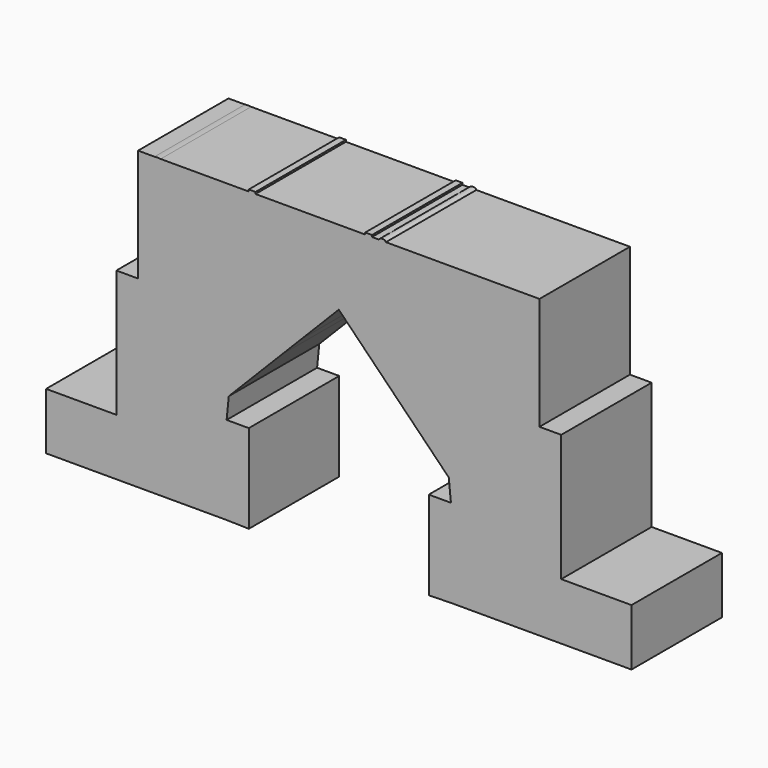
from build123d import *

# Parameters (mm, degrees)
F0_W     = 23.9999517798
F0_H     = 19.3845741451
F0_W_2   = 7.413379848
F0_H_2   = 6.8307565525
F0_W_3   = 2.3086097307
F0_H_3   = 11.162721552
F0_H_4   = 8.4640948573
F0_H_5   = 0.6177287317
F1_DEPTH = 38.608


# Not quite as in the source:
# - a feature names something its author has since deleted; it is built from what else it names


with BuildPart() as f1:
    # F0 (on Front) → F1 (new body)
    with BuildSketch(Plane.XZ):
        with BuildLine():
            Line((-68.5475096107, -12.9382861778), (-12.7116840901, -12.9382861778))
            Line((-12.7116840901, -12.9382861778), (0, 0))
            Line((0, 0), (12.7116840901, -12.9382861778))
            Line((12.7116840901, -12.9382861778), (68.5475096107, -12.9382861778))
            Line((68.5475096107, -12.9382861778), (68.5475096107, 14.3534084782))
            Line((68.5475096107, 14.3534084782), (66.7524240507, 14.3534084782))
            add(Edge.make_bspline(
                [(66.7524240507, 14.3534084782), (66.1189767503, 14.2007931445), (65.3300525788, 14.2007931445)],
                knots=[0.3725049801, 0.3725049801, 0.3725049801, 1, 1, 1], degree=2))
            add(Edge.make_bspline(
                [(65.3300525788, 14.2007931445), (64.6836551195, 14.2007931445), (64.2012071207, 14.3534084782)],
                knots=[0, 0, 0, 0.4664939231, 0.4664939231, 0.4664939231], degree=2))
            Line((64.2012071207, 14.3534084782), (60.0539224702, 14.3534084782))
            Line((60.0539224702, 14.3534084782), (57.7453127395, 14.3534084782))
            Line((57.7453127395, 14.3534084782), (54.5500805939, 14.3534084782))
            Line((54.5500805939, 14.3534084782), (52.2414708632, 14.3534084782))
            Line((52.2414708632, 14.3534084782), (48.6155818967, 14.3534084782))
            add(Edge.make_bspline(
                [(48.6155818967, 14.3534084782), (48.6044206533, 14.3509655306), (48.5932376477, 14.348563547)],
                knots=[0.9837451644, 0.9837451644, 0.9837451644, 1, 1, 1], degree=2))
            add(Edge.make_bspline(
                [(48.5932376477, 14.348563547), (47.9052574131, 14.2007931445), (46.9120465111, 14.2007931445)],
                knots=[0, 0, 0, 1, 1, 1], degree=2))
            add(Edge.make_bspline(
                [(46.9120465111, 14.2007931445), (46.1611803853, 14.2007931445), (45.5308345231, 14.3534084782)],
                knots=[0, 0, 0, 0.3676861883, 0.3676861883, 0.3676861883], degree=2))
            Line((45.5308345231, 14.3534084782), (40.7129570035, 14.3534084782))
            Line((40.7129570035, 14.3534084782), (38.3970798759, 14.3534084782))
            Line((38.3970798759, 14.3534084782), (35.4368268949, 14.3534084782))
            Line((35.4368268949, 14.3534084782), (33.1282171642, 14.3534084782))
            Line((33.1282171642, 14.3534084782), (30.1679641832, 14.3534084782))
            Line((30.1679641832, 14.3534084782), (27.8593544525, 14.3534084782))
            Line((27.8593544525, 14.3534084782), (25.480493219, 14.3534084782))
            Line((25.480493219, 14.3534084782), (23.8695535853, 14.3534084782))
            Line((23.8695535853, 14.3534084782), (21.8041574644, 14.3534084782))
            add(Edge.make_bspline(
                [(21.8041574644, 14.3534084782), (21.2786895623, 14.2007931445), (20.553198159, 14.2007931445)],
                knots=[0.2677635541, 0.2677635541, 0.2677635541, 1, 1, 1], degree=2))
            add(Edge.make_bspline(
                [(20.553198159, 14.2007931445), (19.9832968728, 14.2007931445), (19.5267972582, 14.3534084782)],
                knots=[0, 0, 0, 0.4677071733, 0.4677071733, 0.4677071733], degree=2))
            Line((19.5267972582, 14.3534084782), (16.071636772, 14.3534084782))
            Line((16.071636772, 14.3534084782), (13.7630270413, 14.3534084782))
            Line((13.7630270413, 14.3534084782), (11.3405614268, 14.3534084782))
            Line((11.3405614268, 14.3534084782), (9.0319516961, 14.3534084782))
            Line((9.0319516961, 14.3534084782), (4.3008763508, 14.3534084782))
            Line((4.3008763508, 14.3534084782), (1.9922666201, 14.3534084782))
            Line((1.9922666201, 14.3534084782), (0, 14.3534084782))
            Line((0, 14.3534084782), (-0.3865946134, 14.3534084782))
            Line((-0.3865946134, 14.3534084782), (-1.9975342471, 14.3534084782))
            Line((-1.9975342471, 14.3534084782), (-4.062930368, 14.3534084782))
            add(Edge.make_bspline(
                [(-4.062930368, 14.3534084782), (-4.5883982701, 14.2007931445), (-5.3138896734, 14.2007931445)],
                knots=[0.2677635541, 0.2677635541, 0.2677635541, 1, 1, 1], degree=2))
            add(Edge.make_bspline(
                [(-5.3138896734, 14.2007931445), (-5.8837909596, 14.2007931445), (-6.3402905743, 14.3534084782)],
                knots=[0, 0, 0, 0.4677071733, 0.4677071733, 0.4677071733], degree=2))
            Line((-6.3402905743, 14.3534084782), (-14.5798206492, 14.3534084782))
            Line((-14.5798206492, 14.3534084782), (-16.9271898297, 14.3534084782))
            Line((-16.9271898297, 14.3534084782), (-22.3486678751, 14.3534084782))
            Line((-22.3486678751, 14.3534084782), (-25.0133800512, 14.3534084782))
            Line((-25.0133800512, 14.3534084782), (-28.4435913614, 14.3534084782))
            Line((-28.4435913614, 14.3534084782), (-30.7522010921, 14.3534084782))
            Line((-30.7522010921, 14.3534084782), (-34.3780900586, 14.3534084782))
            add(Edge.make_bspline(
                [(-34.3780900586, 14.3534084782), (-34.389251302, 14.3509655306), (-34.4004343076, 14.348563547)],
                knots=[0.9837451644, 0.9837451644, 0.9837451644, 1, 1, 1], degree=2))
            add(Edge.make_bspline(
                [(-34.4004343076, 14.348563547), (-35.0884145422, 14.2007931445), (-36.0816254441, 14.2007931445)],
                knots=[0, 0, 0, 1, 1, 1], degree=2))
            add(Edge.make_bspline(
                [(-36.0816254441, 14.2007931445), (-36.8324915699, 14.2007931445), (-37.4628374322, 14.3534084782)],
                knots=[0, 0, 0, 0.3676861883, 0.3676861883, 0.3676861883], degree=2))
            Line((-37.4628374322, 14.3534084782), (-43.5374325473, 14.3534084782))
            add(Edge.make_bspline(
                [(-43.5374325473, 14.3534084782), (-43.5485937907, 14.3509655306), (-43.5597767963, 14.348563547)],
                knots=[0.9837451644, 0.9837451644, 0.9837451644, 1, 1, 1], degree=2))
            add(Edge.make_bspline(
                [(-43.5597767963, 14.348563547), (-44.2477570309, 14.2007931445), (-45.2409679328, 14.2007931445)],
                knots=[0, 0, 0, 1, 1, 1], degree=2))
            add(Edge.make_bspline(
                [(-45.2409679328, 14.2007931445), (-45.9918340586, 14.2007931445), (-46.6221799209, 14.3534084782)],
                knots=[0, 0, 0, 0.3676861883, 0.3676861883, 0.3676861883], degree=2))
            Line((-46.6221799209, 14.3534084782), (-53.8019614147, 14.3534084782))
            Line((-53.8019614147, 14.3534084782), (-56.1105711454, 14.3534084782))
            Line((-56.1105711454, 14.3534084782), (-60.4937387393, 14.3534084782))
            add(Edge.make_bspline(
                [(-60.4937387393, 14.3534084782), (-60.5333558618, 14.3471702449), (-60.5727528075, 14.3412961501)],
                knots=[0.958192391, 0.958192391, 0.958192391, 1, 1, 1], degree=2))
            add(Edge.make_bspline(
                [(-60.5727528075, 14.3412961501), (-61.5150919315, 14.2007931445), (-62.4986129711, 14.2007931445)],
                knots=[0, 0, 0, 1, 1, 1], degree=2))
            add(Edge.make_bspline(
                [(-62.4986129711, 14.2007931445), (-63.3049129437, 14.2007931445), (-63.9885935241, 14.3534084782)],
                knots=[0, 0, 0, 0.3218981532, 0.3218981532, 0.3218981532], degree=2))
            Line((-63.9885935241, 14.3534084782), (-68.5475096107, 14.3534084782))
            Line((-68.5475096107, 14.3534084782), (-68.5475096107, -12.9382861778))
        make_face()
        Polygon((-75.9608894587, -56.3228167593), (-75.9608894587, -75.7073909044), (-38.2994301617, -75.7073909044), (-38.2994301617, -45.615144074), (-75.9608894587, -45.615144074), align=None)
        Polygon((75.9608894587, -45.615144074), (38.2994301617, -45.615144074), (38.2994301617, -75.7073909044), (75.9608894587, -75.7073909044), (75.9608894587, -56.3228167593), align=None)
        Polygon((-68.5475096107, -38.2305420935), (-37.5609695911, -38.2305420935), (-19.4228062742, -19.7690427303), (-68.5475096107, -19.7690427303), align=None)
        Polygon((68.5475096107, -19.7690427303), (19.4228062742, -19.7690427303), (37.5609695911, -38.2305420935), (68.5475096107, -38.2305420935), align=None)
        with Locations((-87.9608653486, -66.0151038319)):
            Rectangle(F0_W, F0_H)
        with Locations((87.9608653486, -66.0151038319)):
            Rectangle(F0_W, F0_H)
        Polygon((-68.5475096107, -19.7690427303), (-19.4228062742, -19.7690427303), (-12.7116840901, -12.9382861778), (-68.5475096107, -12.9382861778), align=None)
        Polygon((68.5475096107, -12.9382861778), (12.7116840901, -12.9382861778), (19.4228062742, -19.7690427303), (68.5475096107, -19.7690427303), align=None)
        with BuildLine():
            Line((66.7524240507, 14.3534084782), (68.5475096107, 14.3534084782))
            Line((68.5475096107, 14.3534084782), (68.5475096107, 25.5161300302))
            Line((68.5475096107, 25.5161300302), (16.0930622428, 25.5161300302))
            add(Edge.make_bspline(
                [(16.0930622428, 25.5161300302), (16.1782252591, 25.2987930153), (16.1782252591, 25.0049897855)],
                knots=[0.7397366426, 0.7397366426, 0.7397366426, 1, 1, 1], degree=2))
            add(Edge.make_bspline(
                [(16.1782252591, 25.0049897855), (16.1782252591, 24.467202419), (15.864515962, 24.1680279156)],
                knots=[0, 0, 0, 1, 1, 1], degree=2))
            add(Edge.make_bspline(
                [(15.864515962, 24.1680279156), (15.5508066649, 23.8688534122), (14.9209656051, 23.8688534122)],
                knots=[0, 0, 0, 1, 1, 1], degree=2))
            add(Edge.make_bspline(
                [(14.9209656051, 23.8688534122), (13.6637059511, 23.8688534122), (13.6637059511, 25.0049897855)],
                knots=[0, 0, 0, 1, 1, 1], degree=2))
            add(Edge.make_bspline(
                [(13.6637059511, 25.0049897855), (13.6637059511, 25.2987930153), (13.7488689674, 25.5161300302)],
                knots=[0, 0, 0, 0.2602633574, 0.2602633574, 0.2602633574], degree=2))
            Line((13.7488689674, 25.5161300302), (11.3405614268, 25.5161300302))
            Line((11.3405614268, 25.5161300302), (11.3405614268, 14.3534084782))
            Line((11.3405614268, 14.3534084782), (13.7630270413, 14.3534084782))
            Line((13.7630270413, 14.3534084782), (13.7630270413, 22.8175033355))
            Line((13.7630270413, 22.8175033355), (16.071636772, 22.8175033355))
            Line((16.071636772, 22.8175033355), (16.071636772, 14.3534084782))
            Line((16.071636772, 14.3534084782), (19.5267972582, 14.3534084782))
            add(Edge.make_bspline(
                [(19.5267972582, 14.3534084782), (19.0072596413, 14.5270984535), (18.6346053922, 14.8984632415)],
                knots=[0.4677071733, 0.4677071733, 0.4677071733, 1, 1, 1], degree=2))
            add(Edge.make_bspline(
                [(18.6346053922, 14.8984632415), (17.9345128296, 15.5961333385), (17.9345128296, 16.8824625798)],
                knots=[0, 0, 0, 1, 1, 1], degree=2))
            add(Edge.make_bspline(
                [(17.9345128296, 16.8824625798), (17.9345128296, 18.2293534615), (18.8768519537, 18.8688843838)],
                knots=[0, 0, 0, 1, 1, 1], degree=2))
            add(Edge.make_bspline(
                [(18.8768519537, 18.8688843838), (19.8191910778, 19.508415306), (21.7184041196, 19.5762443432)],
                knots=[0, 0, 0, 1, 1, 1], degree=2))
            Line((21.7184041196, 19.5762443432), (23.1888407476, 19.6222711899))
            Line((23.1888407476, 19.6222711899), (23.1888407476, 19.9929084289))
            add(Edge.make_bspline(
                [(23.1888407476, 19.9929084289), (23.1888407476, 21.2792376703), (21.8710194533, 21.2792376703)],
                knots=[0, 0, 0, 1, 1, 1], degree=2))
            add(Edge.make_bspline(
                [(21.8710194533, 21.2792376703), (20.8560063608, 21.2792376703), (19.4848908229, 20.6663538698)],
                knots=[0, 0, 0, 1, 1, 1], degree=2))
            Line((19.4848908229, 20.6663538698), (18.7218141544, 22.2264217256))
            add(Edge.make_bspline(
                [(18.7218141544, 22.2264217256), (20.1825609199, 22.9919208598), (21.960650681, 22.9919208598)],
                knots=[0, 0, 0, 1, 1, 1], degree=2))
            add(Edge.make_bspline(
                [(21.960650681, 22.9919208598), (23.6636440081, 22.9919208598), (24.5720686136, 22.2494351489)],
                knots=[0, 0, 0, 1, 1, 1], degree=2))
            add(Edge.make_bspline(
                [(24.5720686136, 22.2494351489), (25.480493219, 21.506949438), (25.480493219, 19.9929084289)],
                knots=[0, 0, 0, 1, 1, 1], degree=2))
            Line((25.480493219, 19.9929084289), (25.480493219, 14.3534084782))
            Line((25.480493219, 14.3534084782), (27.8593544525, 14.3534084782))
            Line((27.8593544525, 14.3534084782), (27.8593544525, 22.8175033355))
            Line((27.8593544525, 22.8175033355), (29.6229094199, 22.8175033355))
            Line((29.6229094199, 22.8175033355), (29.9329850186, 21.7346612058))
            Line((29.9329850186, 21.7346612058), (30.0613756962, 21.7346612058))
            add(Edge.make_bspline(
                [(30.0613756962, 21.7346612058), (30.4029433478, 22.3184754189), (31.0461079685, 22.6467195097)],
                knots=[0, 0, 0, 1, 1, 1], degree=2))
            add(Edge.make_bspline(
                [(31.0461079685, 22.6467195097), (31.6892725892, 22.9749636005), (32.5226007606, 22.9749636005)],
                knots=[0, 0, 0, 1, 1, 1], degree=2))
            add(Edge.make_bspline(
                [(32.5226007606, 22.9749636005), (34.4218138024, 22.9749636005), (35.0976817089, 21.7346612058)],
                knots=[0, 0, 0, 1, 1, 1], degree=2))
            Line((35.0976817089, 21.7346612058), (35.3011688205, 21.7346612058))
            add(Edge.make_bspline(
                [(35.3011688205, 21.7346612058), (35.6427364722, 22.3257428158), (36.3040695849, 22.6503532081)],
                knots=[0, 0, 0, 1, 1, 1], degree=2))
            add(Edge.make_bspline(
                [(36.3040695849, 22.6503532081), (36.9654026977, 22.9749636005), (37.7987308691, 22.9749636005)],
                knots=[0, 0, 0, 1, 1, 1], degree=2))
            add(Edge.make_bspline(
                [(37.7987308691, 22.9749636005), (39.2376754442, 22.9749636005), (39.9753162238, 22.2373228208)],
                knots=[0, 0, 0, 1, 1, 1], degree=2))
            add(Edge.make_bspline(
                [(39.9753162238, 22.2373228208), (40.7129570035, 21.4996820412), (40.7129570035, 19.8717851482)],
                knots=[0, 0, 0, 1, 1, 1], degree=2))
            Line((40.7129570035, 19.8717851482), (40.7129570035, 14.3534084782))
            Line((40.7129570035, 14.3534084782), (45.5308345231, 14.3534084782))
            add(Edge.make_bspline(
                [(45.5308345231, 14.3534084782), (44.4468221027, 14.6158626755), (43.7192368311, 15.3296621209)],
                knots=[0.3676861883, 0.3676861883, 0.3676861883, 1, 1, 1], degree=2))
            add(Edge.make_bspline(
                [(43.7192368311, 15.3296621209), (42.5685656642, 16.4585310973), (42.5685656642, 18.5248942665)],
                knots=[0, 0, 0, 1, 1, 1], degree=2))
            add(Edge.make_bspline(
                [(42.5685656642, 18.5248942665), (42.5685656642, 20.6518190761), (43.632028069, 21.8133913383)],
                knots=[0, 0, 0, 1, 1, 1], degree=2))
            add(Edge.make_bspline(
                [(43.632028069, 21.8133913383), (44.6954904738, 22.9749636005), (46.5729013251, 22.9749636005)],
                knots=[0, 0, 0, 1, 1, 1], degree=2))
            add(Edge.make_bspline(
                [(46.5729013251, 22.9749636005), (48.3655258799, 22.9749636005), (49.3647929459, 21.9538943439)],
                knots=[0, 0, 0, 1, 1, 1], degree=2))
            add(Edge.make_bspline(
                [(49.3647929459, 21.9538943439), (50.3640600119, 20.9328250874), (50.3640600119, 19.1305106701)],
                knots=[0, 0, 0, 1, 1, 1], degree=2))
            Line((50.3640600119, 19.1305106701), (50.3640600119, 18.0089090906))
            Line((50.3640600119, 18.0089090906), (44.9062449823, 18.0089090906))
            add(Edge.make_bspline(
                [(44.9062449823, 18.0089090906), (44.9450044321, 17.0253880511), (45.4900591954, 16.473065891)],
                knots=[0, 0, 0, 1, 1, 1], degree=2))
            add(Edge.make_bspline(
                [(45.4900591954, 16.473065891), (46.0351139587, 15.9207437308), (47.0186349982, 15.9207437308)],
                knots=[0, 0, 0, 1, 1, 1], degree=2))
            add(Edge.make_bspline(
                [(47.0186349982, 15.9207437308), (47.7841341324, 15.9207437308), (48.4648469701, 16.0794152286)],
                knots=[0, 0, 0, 1, 1, 1], degree=2))
            add(Edge.make_bspline(
                [(48.4648469701, 16.0794152286), (49.1455598078, 16.2380867263), (49.8868342858, 16.5869217748)],
                knots=[0, 0, 0, 1, 1, 1], degree=2))
            Line((49.8868342858, 16.5869217748), (49.8868342858, 14.7991421513))
            add(Edge.make_bspline(
                [(49.8868342858, 14.7991421513), (49.2910620773, 14.501256047), (48.6155818967, 14.3534084782)],
                knots=[0, 0, 0, 0.9837451644, 0.9837451644, 0.9837451644], degree=2))
            Line((48.6155818967, 14.3534084782), (52.2414708632, 14.3534084782))
            Line((52.2414708632, 14.3534084782), (52.2414708632, 22.8175033355))
            Line((52.2414708632, 22.8175033355), (54.0050258306, 22.8175033355))
            Line((54.0050258306, 22.8175033355), (54.3151014293, 21.7346612058))
            Line((54.3151014293, 21.7346612058), (54.4434921069, 21.7346612058))
            add(Edge.make_bspline(
                [(54.4434921069, 21.7346612058), (54.8310866052, 22.3475450063), (55.5081657445, 22.6612543034)],
                knots=[0, 0, 0, 1, 1, 1], degree=2))
            add(Edge.make_bspline(
                [(55.5081657445, 22.6612543034), (56.1852448837, 22.9749636005), (57.0476426425, 22.9749636005)],
                knots=[0, 0, 0, 1, 1, 1], degree=2))
            add(Edge.make_bspline(
                [(57.0476426425, 22.9749636005), (58.5253466674, 22.9749636005), (59.2896345688, 22.1767611805)],
                knots=[0, 0, 0, 1, 1, 1], degree=2))
            add(Edge.make_bspline(
                [(59.2896345688, 22.1767611805), (60.0539224702, 21.3785587605), (60.0539224702, 19.8717851482)],
                knots=[0, 0, 0, 1, 1, 1], degree=2))
            Line((60.0539224702, 19.8717851482), (60.0539224702, 14.3534084782))
            Line((60.0539224702, 14.3534084782), (64.2012071207, 14.3534084782))
            add(Edge.make_bspline(
                [(64.2012071207, 14.3534084782), (63.6494551548, 14.5279471033), (63.3121387218, 14.9020969399)],
                knots=[0.4664939231, 0.4664939231, 0.4664939231, 1, 1, 1], degree=2))
            add(Edge.make_bspline(
                [(63.3121387218, 14.9020969399), (62.6798751964, 15.6034007353), (62.6798751964, 17.0035858605)],
                knots=[0, 0, 0, 1, 1, 1], degree=2))
            Line((62.6798751964, 17.0035858605), (62.6798751964, 21.0830179555))
            Line((62.6798751964, 21.0830179555), (61.5752308762, 21.0830179555))
            Line((61.5752308762, 21.0830179555), (61.5752308762, 22.0592715982))
            Line((61.5752308762, 22.0592715982), (62.8470253238, 22.8320381292))
            Line((62.8470253238, 22.8320381292), (63.5132033678, 24.6198177528))
            Line((63.5132033678, 24.6198177528), (64.9884849271, 24.6198177528))
            Line((64.9884849271, 24.6198177528), (64.9884849271, 22.8175033355))
            Line((64.9884849271, 22.8175033355), (67.3576562982, 22.8175033355))
            Line((67.3576562982, 22.8175033355), (67.3576562982, 21.0830179555))
            Line((67.3576562982, 21.0830179555), (64.9884849271, 21.0830179555))
            Line((64.9884849271, 21.0830179555), (64.9884849271, 17.0035858605))
            add(Edge.make_bspline(
                [(64.9884849271, 17.0035858605), (64.9884849271, 16.5118253408), (65.2646460072, 16.2768461762)],
                knots=[0, 0, 0, 1, 1, 1], degree=2))
            add(Edge.make_bspline(
                [(65.2646460072, 16.2768461762), (65.5408070872, 16.0418670116), (65.9962306228, 16.0418670116)],
                knots=[0, 0, 0, 1, 1, 1], degree=2))
            add(Edge.make_bspline(
                [(65.9962306228, 16.0418670116), (66.6018470264, 16.0418670116), (67.4497099915, 16.3059157635)],
                knots=[0, 0, 0, 1, 1, 1], degree=2))
            Line((67.4497099915, 16.3059157635), (67.4497099915, 14.5883876428))
            add(Edge.make_bspline(
                [(67.4497099915, 14.5883876428), (67.1284625315, 14.4440067619), (66.7524240507, 14.3534084782)],
                knots=[0, 0, 0, 0.3725049801, 0.3725049801, 0.3725049801], degree=2))
        make_face()
        Polygon((-75.9608894587, -38.2305420935), (-75.9608894587, -45.615144074), (-38.2994301617, -45.615144074), (-37.5609695911, -38.2305420935), (-68.5475096107, -38.2305420935), (-73.0070546269, -38.2305420935), align=None)
        Polygon((68.5475096107, -38.2305420935), (37.5609695911, -38.2305420935), (38.2994301617, -45.615144074), (75.9608894587, -45.615144074), (75.9608894587, -38.2305420935), (73.0070546269, -38.2305420935), align=None)
        with BuildLine():
            Line((0, 25.5161300302), (-28.4435913614, 25.5161300302))
            Line((-28.4435913614, 25.5161300302), (-28.4435913614, 20.8795308439))
            Line((-28.4435913614, 20.8795308439), (-28.5647146421, 18.9560931459))
            Line((-28.5647146421, 18.9560931459), (-28.5332225891, 18.9560931459))
            Line((-28.5332225891, 18.9560931459), (-27.5278993591, 20.2424223872))
            Line((-27.5278993591, 20.2424223872), (-25.158727988, 22.8175033355))
            Line((-25.158727988, 22.8175033355), (-22.5545774524, 22.8175033355))
            Line((-22.5545774524, 22.8175033355), (-25.9145372598, 19.1450454638))
            Line((-25.9145372598, 19.1450454638), (-22.3486678751, 14.3534084782))
            Line((-22.3486678751, 14.3534084782), (-16.9271898297, 14.3534084782))
            Line((-16.9271898297, 14.3534084782), (-16.9271898297, 25.4216538712))
            Line((-16.9271898297, 25.4216538712), (-13.392812498, 25.4216538712))
            add(Edge.make_bspline(
                [(-13.392812498, 25.4216538712), (-11.3773211067, 25.4216538712), (-10.3296047284, 24.5544111812)],
                knots=[0, 0, 0, 1, 1, 1], degree=2))
            add(Edge.make_bspline(
                [(-10.3296047284, 24.5544111812), (-9.2818883501, 23.6871684912), (-9.2818883501, 21.9696403704)],
                knots=[0, 0, 0, 1, 1, 1], degree=2))
            add(Edge.make_bspline(
                [(-9.2818883501, 21.9696403704), (-9.2818883501, 20.1818607469), (-10.3986449984, 19.2358879244)],
                knots=[0, 0, 0, 1, 1, 1], degree=2))
            add(Edge.make_bspline(
                [(-10.3986449984, 19.2358879244), (-11.5154016467, 18.2899151019), (-13.5744974191, 18.2899151019)],
                knots=[0, 0, 0, 1, 1, 1], degree=2))
            Line((-13.5744974191, 18.2899151019), (-14.5798206492, 18.2899151019))
            Line((-14.5798206492, 18.2899151019), (-14.5798206492, 14.3534084782))
            Line((-14.5798206492, 14.3534084782), (-6.3402905743, 14.3534084782))
            add(Edge.make_bspline(
                [(-6.3402905743, 14.3534084782), (-6.8598281911, 14.5270984535), (-7.2324824402, 14.8984632415)],
                knots=[0.4677071733, 0.4677071733, 0.4677071733, 1, 1, 1], degree=2))
            add(Edge.make_bspline(
                [(-7.2324824402, 14.8984632415), (-7.9325750028, 15.5961333385), (-7.9325750028, 16.8824625798)],
                knots=[0, 0, 0, 1, 1, 1], degree=2))
            add(Edge.make_bspline(
                [(-7.9325750028, 16.8824625798), (-7.9325750028, 18.2293534615), (-6.9902358787, 18.8688843838)],
                knots=[0, 0, 0, 1, 1, 1], degree=2))
            add(Edge.make_bspline(
                [(-6.9902358787, 18.8688843838), (-6.0478967547, 19.508415306), (-4.1486837128, 19.5762443432)],
                knots=[0, 0, 0, 1, 1, 1], degree=2))
            Line((-4.1486837128, 19.5762443432), (-2.6782470848, 19.6222711899))
            Line((-2.6782470848, 19.6222711899), (-2.6782470848, 19.9929084289))
            add(Edge.make_bspline(
                [(-2.6782470848, 19.9929084289), (-2.6782470848, 21.2792376703), (-3.9960683791, 21.2792376703)],
                knots=[0, 0, 0, 1, 1, 1], degree=2))
            add(Edge.make_bspline(
                [(-3.9960683791, 21.2792376703), (-5.0110814716, 21.2792376703), (-6.3821970095, 20.6663538698)],
                knots=[0, 0, 0, 1, 1, 1], degree=2))
            Line((-6.3821970095, 20.6663538698), (-7.1452736781, 22.2264217256))
            add(Edge.make_bspline(
                [(-7.1452736781, 22.2264217256), (-5.6845269125, 22.9919208598), (-3.9064371514, 22.9919208598)],
                knots=[0, 0, 0, 1, 1, 1], degree=2))
            add(Edge.make_bspline(
                [(-3.9064371514, 22.9919208598), (-2.2034438243, 22.9919208598), (-1.2950192189, 22.2494351489)],
                knots=[0, 0, 0, 1, 1, 1], degree=2))
            add(Edge.make_bspline(
                [(-1.2950192189, 22.2494351489), (-0.3865946134, 21.506949438), (-0.3865946134, 19.9929084289)],
                knots=[0, 0, 0, 1, 1, 1], degree=2))
            Line((-0.3865946134, 19.9929084289), (-0.3865946134, 14.3534084782))
            Line((-0.3865946134, 14.3534084782), (0, 14.3534084782))
            Line((0, 14.3534084782), (1.9922666201, 14.3534084782))
            Line((1.9922666201, 14.3534084782), (1.9922666201, 22.8175033355))
            Line((1.9922666201, 22.8175033355), (3.7412867938, 22.8175033355))
            Line((3.7412867938, 22.8175033355), (4.0828544455, 21.3930935542))
            Line((4.0828544455, 21.3930935542), (4.1942878638, 21.3930935542))
            add(Edge.make_bspline(
                [(4.1942878638, 21.3930935542), (4.5891497589, 22.1052984448), (5.2589615014, 22.5401310227)],
                knots=[0, 0, 0, 1, 1, 1], degree=2))
            add(Edge.make_bspline(
                [(5.2589615014, 22.5401310227), (5.9287732438, 22.9749636005), (6.7160745685, 22.9749636005)],
                knots=[0, 0, 0, 1, 1, 1], degree=2))
            add(Edge.make_bspline(
                [(6.7160745685, 22.9749636005), (7.1860328978, 22.9749636005), (7.4961084964, 22.9071345633)],
                knots=[0, 0, 0, 1, 1, 1], degree=2))
            Line((7.4961084964, 22.9071345633), (7.3216909722, 20.7438727694))
            add(Edge.make_bspline(
                [(7.3216909722, 20.7438727694), (7.0406849609, 20.8189692035), (6.6409781345, 20.8189692035)],
                knots=[0, 0, 0, 1, 1, 1], degree=2))
            add(Edge.make_bspline(
                [(6.6409781345, 20.8189692035), (5.5363338142, 20.8189692035), (4.9186050825, 20.2509010169)],
                knots=[0, 0, 0, 1, 1, 1], degree=2))
            add(Edge.make_bspline(
                [(4.9186050825, 20.2509010169), (4.3008763508, 19.6828328303), (4.3008763508, 18.6605523409)],
                knots=[0, 0, 0, 1, 1, 1], degree=2))
            Line((4.3008763508, 18.6605523409), (4.3008763508, 14.3534084782))
            Line((4.3008763508, 14.3534084782), (9.0319516961, 14.3534084782))
            Line((9.0319516961, 14.3534084782), (9.0319516961, 25.5161300302))
            Line((9.0319516961, 25.5161300302), (0, 25.5161300302))
        make_face()
        Polygon((-38.2994301617, -45.615144074), (-38.2994301617, -75.7073909044), (-30.7302121073, -75.892008841), (-30.7302121073, -45.615144074), align=None)
        Polygon((38.2994301617, -75.7073909044), (38.2994301617, -45.615144074), (30.7302121073, -45.615144074), (30.7302121073, -75.892008841), align=None)
        with BuildLine():
            add(Edge.make_bspline(
                [(-58.5621063474, 14.8306342043), (-59.585750308, 14.4963831151), (-60.4937387393, 14.3534084782)],
                knots=[0, 0, 0, 0.958192391, 0.958192391, 0.958192391], degree=2))
            Line((-60.4937387393, 14.3534084782), (-56.1105711454, 14.3534084782))
            Line((-56.1105711454, 14.3534084782), (-56.1105711454, 22.8175033355))
            Line((-56.1105711454, 22.8175033355), (-54.3615509717, 22.8175033355))
            Line((-54.3615509717, 22.8175033355), (-54.0199833201, 21.3930935542))
            Line((-54.0199833201, 21.3930935542), (-53.9085499018, 21.3930935542))
            add(Edge.make_bspline(
                [(-53.9085499018, 21.3930935542), (-53.5136880066, 22.1052984448), (-52.8438762642, 22.5401310227)],
                knots=[0, 0, 0, 1, 1, 1], degree=2))
            add(Edge.make_bspline(
                [(-52.8438762642, 22.5401310227), (-52.1740645218, 22.9749636005), (-51.386763197, 22.9749636005)],
                knots=[0, 0, 0, 1, 1, 1], degree=2))
            add(Edge.make_bspline(
                [(-51.386763197, 22.9749636005), (-50.9168048678, 22.9749636005), (-50.6067292691, 22.9071345633)],
                knots=[0, 0, 0, 1, 1, 1], degree=2))
            Line((-50.6067292691, 22.9071345633), (-50.7811467934, 20.7438727694))
            add(Edge.make_bspline(
                [(-50.7811467934, 20.7438727694), (-51.0621528047, 20.8189692035), (-51.4618596311, 20.8189692035)],
                knots=[0, 0, 0, 1, 1, 1], degree=2))
            add(Edge.make_bspline(
                [(-51.4618596311, 20.8189692035), (-52.5665039513, 20.8189692035), (-53.184232683, 20.2509010169)],
                knots=[0, 0, 0, 1, 1, 1], degree=2))
            add(Edge.make_bspline(
                [(-53.184232683, 20.2509010169), (-53.8019614147, 19.6828328303), (-53.8019614147, 18.6605523409)],
                knots=[0, 0, 0, 1, 1, 1], degree=2))
            Line((-53.8019614147, 18.6605523409), (-53.8019614147, 14.3534084782))
            Line((-53.8019614147, 14.3534084782), (-46.6221799209, 14.3534084782))
            add(Edge.make_bspline(
                [(-46.6221799209, 14.3534084782), (-47.7061923412, 14.6158626755), (-48.4337776128, 15.3296621209)],
                knots=[0.3676861883, 0.3676861883, 0.3676861883, 1, 1, 1], degree=2))
            add(Edge.make_bspline(
                [(-48.4337776128, 15.3296621209), (-49.5844487798, 16.4585310973), (-49.5844487798, 18.5248942665)],
                knots=[0, 0, 0, 1, 1, 1], degree=2))
            add(Edge.make_bspline(
                [(-49.5844487798, 18.5248942665), (-49.5844487798, 20.6518190761), (-48.520986375, 21.8133913383)],
                knots=[0, 0, 0, 1, 1, 1], degree=2))
            add(Edge.make_bspline(
                [(-48.520986375, 21.8133913383), (-47.4575239702, 22.9749636005), (-45.5801131189, 22.9749636005)],
                knots=[0, 0, 0, 1, 1, 1], degree=2))
            add(Edge.make_bspline(
                [(-45.5801131189, 22.9749636005), (-43.7874885641, 22.9749636005), (-42.7882214981, 21.9538943439)],
                knots=[0, 0, 0, 1, 1, 1], degree=2))
            add(Edge.make_bspline(
                [(-42.7882214981, 21.9538943439), (-41.7889544321, 20.9328250874), (-41.7889544321, 19.1305106701)],
                knots=[0, 0, 0, 1, 1, 1], degree=2))
            Line((-41.7889544321, 19.1305106701), (-41.7889544321, 18.0089090906))
            Line((-41.7889544321, 18.0089090906), (-47.2467694617, 18.0089090906))
            add(Edge.make_bspline(
                [(-47.2467694617, 18.0089090906), (-47.2080100119, 17.0253880511), (-46.6629552486, 16.473065891)],
                knots=[0, 0, 0, 1, 1, 1], degree=2))
            add(Edge.make_bspline(
                [(-46.6629552486, 16.473065891), (-46.1179004853, 15.9207437308), (-45.1343794458, 15.9207437308)],
                knots=[0, 0, 0, 1, 1, 1], degree=2))
            add(Edge.make_bspline(
                [(-45.1343794458, 15.9207437308), (-44.3688803116, 15.9207437308), (-43.6881674739, 16.0794152286)],
                knots=[0, 0, 0, 1, 1, 1], degree=2))
            add(Edge.make_bspline(
                [(-43.6881674739, 16.0794152286), (-43.0074546362, 16.2380867263), (-42.2661801581, 16.5869217748)],
                knots=[0, 0, 0, 1, 1, 1], degree=2))
            Line((-42.2661801581, 16.5869217748), (-42.2661801581, 14.7991421513))
            add(Edge.make_bspline(
                [(-42.2661801581, 14.7991421513), (-42.8619523667, 14.501256047), (-43.5374325473, 14.3534084782)],
                knots=[0, 0, 0, 0.9837451644, 0.9837451644, 0.9837451644], degree=2))
            Line((-43.5374325473, 14.3534084782), (-37.4628374322, 14.3534084782))
            add(Edge.make_bspline(
                [(-37.4628374322, 14.3534084782), (-38.5468498525, 14.6158626755), (-39.2744351241, 15.3296621209)],
                knots=[0.3676861883, 0.3676861883, 0.3676861883, 1, 1, 1], degree=2))
            add(Edge.make_bspline(
                [(-39.2744351241, 15.3296621209), (-40.4251062911, 16.4585310973), (-40.4251062911, 18.5248942665)],
                knots=[0, 0, 0, 1, 1, 1], degree=2))
            add(Edge.make_bspline(
                [(-40.4251062911, 18.5248942665), (-40.4251062911, 20.6518190761), (-39.3616438863, 21.8133913383)],
                knots=[0, 0, 0, 1, 1, 1], degree=2))
            add(Edge.make_bspline(
                [(-39.3616438863, 21.8133913383), (-38.2981814815, 22.9749636005), (-36.4207706302, 22.9749636005)],
                knots=[0, 0, 0, 1, 1, 1], degree=2))
            add(Edge.make_bspline(
                [(-36.4207706302, 22.9749636005), (-34.6281460754, 22.9749636005), (-33.6288790094, 21.9538943439)],
                knots=[0, 0, 0, 1, 1, 1], degree=2))
            add(Edge.make_bspline(
                [(-33.6288790094, 21.9538943439), (-32.6296119434, 20.9328250874), (-32.6296119434, 19.1305106701)],
                knots=[0, 0, 0, 1, 1, 1], degree=2))
            Line((-32.6296119434, 19.1305106701), (-32.6296119434, 18.0089090906))
            Line((-32.6296119434, 18.0089090906), (-38.087426973, 18.0089090906))
            add(Edge.make_bspline(
                [(-38.087426973, 18.0089090906), (-38.0486675232, 17.0253880511), (-37.5036127599, 16.473065891)],
                knots=[0, 0, 0, 1, 1, 1], degree=2))
            add(Edge.make_bspline(
                [(-37.5036127599, 16.473065891), (-36.9585579966, 15.9207437308), (-35.9750369571, 15.9207437308)],
                knots=[0, 0, 0, 1, 1, 1], degree=2))
            add(Edge.make_bspline(
                [(-35.9750369571, 15.9207437308), (-35.2095378229, 15.9207437308), (-34.5288249852, 16.0794152286)],
                knots=[0, 0, 0, 1, 1, 1], degree=2))
            add(Edge.make_bspline(
                [(-34.5288249852, 16.0794152286), (-33.8481121475, 16.2380867263), (-33.1068376694, 16.5869217748)],
                knots=[0, 0, 0, 1, 1, 1], degree=2))
            Line((-33.1068376694, 16.5869217748), (-33.1068376694, 14.7991421513))
            add(Edge.make_bspline(
                [(-33.1068376694, 14.7991421513), (-33.702609878, 14.501256047), (-34.3780900586, 14.3534084782)],
                knots=[0, 0, 0, 0.9837451644, 0.9837451644, 0.9837451644], degree=2))
            Line((-34.3780900586, 14.3534084782), (-30.7522010921, 14.3534084782))
            Line((-30.7522010921, 14.3534084782), (-30.7522010921, 25.5161300302))
            Line((-30.7522010921, 25.5161300302), (-60.8378446787, 25.5161300302))
            add(Edge.make_bspline(
                [(-60.8378446787, 25.5161300302), (-59.6773347897, 25.3720535423), (-58.5766411411, 24.8984012984)],
                knots=[0.3041820021, 0.3041820021, 0.3041820021, 1, 1, 1], degree=2))
            Line((-58.5766411411, 24.8984012984), (-59.356675069, 23.0209904471))
            add(Edge.make_bspline(
                [(-59.356675069, 23.0209904471), (-60.5679078762, 23.6266068508), (-61.8784617737, 23.6266068508)],
                knots=[0, 0, 0, 1, 1, 1], degree=2))
            add(Edge.make_bspline(
                [(-61.8784617737, 23.6266068508), (-63.3997701797, 23.6266068508), (-64.315462182, 22.6043263614)],
                knots=[0, 0, 0, 1, 1, 1], degree=2))
            add(Edge.make_bspline(
                [(-64.315462182, 22.6043263614), (-65.2311541843, 21.5820458721), (-65.2311541843, 19.8572503545)],
                knots=[0, 0, 0, 1, 1, 1], degree=2))
            add(Edge.make_bspline(
                [(-65.2311541843, 19.8572503545), (-65.2311541843, 18.0549359373), (-64.4935134047, 17.1053294164)],
                knots=[0, 0, 0, 1, 1, 1], degree=2))
            add(Edge.make_bspline(
                [(-64.4935134047, 17.1053294164), (-63.755872625, 16.1557228954), (-62.348420103, 16.1557228954)],
                knots=[0, 0, 0, 1, 1, 1], degree=2))
            add(Edge.make_bspline(
                [(-62.348420103, 16.1557228954), (-61.6119905561, 16.1557228954), (-60.8561812844, 16.3059157635)],
                knots=[0, 0, 0, 1, 1, 1], degree=2))
            Line((-60.8561812844, 16.3059157635), (-60.8561812844, 18.6145254942))
            Line((-60.8561812844, 18.6145254942), (-62.9540365066, 18.6145254942))
            Line((-62.9540365066, 18.6145254942), (-62.9540365066, 20.5694552452))
            Line((-62.9540365066, 20.5694552452), (-58.5621063474, 20.5694552452))
            Line((-58.5621063474, 20.5694552452), (-58.5621063474, 14.8306342043))
        make_face()
        Polygon((-75.9608894587, -19.7690427303), (-75.9608894587, -38.2305420935), (-73.0070546269, -38.2305420935), (-68.5475096107, -38.2305420935), (-68.5475096107, -19.7690427303), align=None)
        Polygon((75.9608894587, -19.7690427303), (68.5475096107, -19.7690427303), (68.5475096107, -38.2305420935), (73.0070546269, -38.2305420935), (75.9608894587, -38.2305420935), align=None)
        with BuildLine():
            Line((38.3970798759, 14.3534084782), (40.7129570035, 14.3534084782))
            Line((40.7129570035, 14.3534084782), (40.7129570035, 19.8717851482))
            add(Edge.make_bspline(
                [(39.9753162238, 22.2373228208), (40.7129570035, 21.4996820412), (40.7129570035, 19.8717851482)],
                knots=[0, 0, 0, 1, 1, 1], degree=2))
            add(Edge.make_bspline(
                [(37.7987308691, 22.9749636005), (39.2376754442, 22.9749636005), (39.9753162238, 22.2373228208)],
                knots=[0, 0, 0, 1, 1, 1], degree=2))
            add(Edge.make_bspline(
                [(36.3040695849, 22.6503532081), (36.9654026977, 22.9749636005), (37.7987308691, 22.9749636005)],
                knots=[0, 0, 0, 1, 1, 1], degree=2))
            add(Edge.make_bspline(
                [(35.3011688205, 21.7346612058), (35.6427364722, 22.3257428158), (36.3040695849, 22.6503532081)],
                knots=[0, 0, 0, 1, 1, 1], degree=2))
            Line((35.3011688205, 21.7346612058), (35.0976817089, 21.7346612058))
            add(Edge.make_bspline(
                [(32.5226007606, 22.9749636005), (34.4218138024, 22.9749636005), (35.0976817089, 21.7346612058)],
                knots=[0, 0, 0, 1, 1, 1], degree=2))
            add(Edge.make_bspline(
                [(31.0461079685, 22.6467195097), (31.6892725892, 22.9749636005), (32.5226007606, 22.9749636005)],
                knots=[0, 0, 0, 1, 1, 1], degree=2))
            add(Edge.make_bspline(
                [(30.0613756962, 21.7346612058), (30.4029433478, 22.3184754189), (31.0461079685, 22.6467195097)],
                knots=[0, 0, 0, 1, 1, 1], degree=2))
            Line((30.0613756962, 21.7346612058), (29.9329850186, 21.7346612058))
            Line((29.9329850186, 21.7346612058), (29.6229094199, 22.8175033355))
            Line((29.6229094199, 22.8175033355), (27.8593544525, 22.8175033355))
            Line((27.8593544525, 22.8175033355), (27.8593544525, 14.3534084782))
            Line((27.8593544525, 14.3534084782), (30.1679641832, 14.3534084782))
            Line((30.1679641832, 14.3534084782), (30.1679641832, 18.3359419486))
            add(Edge.make_bspline(
                [(30.5688822424, 20.4774015518), (30.1679641832, 19.8257583015), (30.1679641832, 18.3359419486)],
                knots=[0, 0, 0, 1, 1, 1], degree=2))
            add(Edge.make_bspline(
                [(31.8564227166, 21.1290448022), (30.9698003016, 21.1290448022), (30.5688822424, 20.4774015518)],
                knots=[0, 0, 0, 1, 1, 1], degree=2))
            add(Edge.make_bspline(
                [(32.821775264, 20.671198801), (32.5153333637, 21.1290448022), (31.8564227166, 21.1290448022)],
                knots=[0, 0, 0, 1, 1, 1], degree=2))
            add(Edge.make_bspline(
                [(33.1282171642, 19.2976607975), (33.1282171642, 20.2133527999), (32.821775264, 20.671198801)],
                knots=[0, 0, 0, 1, 1, 1], degree=2))
            Line((33.1282171642, 19.2976607975), (33.1282171642, 14.3534084782))
            Line((33.1282171642, 14.3534084782), (35.4368268949, 14.3534084782))
            Line((35.4368268949, 14.3534084782), (35.4368268949, 18.5999907005))
            add(Edge.make_bspline(
                [(35.857124679, 20.5234283985), (35.4368268949, 19.9178119949), (35.4368268949, 18.5999907005)],
                knots=[0, 0, 0, 1, 1, 1], degree=2))
            add(Edge.make_bspline(
                [(37.1252854283, 21.1290448022), (36.2774224632, 21.1290448022), (35.857124679, 20.5234283985)],
                knots=[0, 0, 0, 1, 1, 1], degree=2))
            add(Edge.make_bspline(
                [(38.0906379757, 20.671198801), (37.7841960754, 21.1290448022), (37.1252854283, 21.1290448022)],
                knots=[0, 0, 0, 1, 1, 1], degree=2))
            add(Edge.make_bspline(
                [(38.3970798759, 19.2976607975), (38.3970798759, 20.2133527999), (38.0906379757, 20.671198801)],
                knots=[0, 0, 0, 1, 1, 1], degree=2))
            Line((38.3970798759, 19.2976607975), (38.3970798759, 14.3534084782))
        make_face()
        with BuildLine():
            add(Edge.make_bspline(
                [(-63.9885935241, 14.3534084782), (-65.4288163383, 14.6749037667), (-66.3248974093, 15.6736522381)],
                knots=[0.3218981532, 0.3218981532, 0.3218981532, 1, 1, 1], degree=2))
            Line((-63.9885935241, 14.3534084782), (-60.4937387393, 14.3534084782))
            add(Edge.make_bspline(
                [(-58.5621063474, 14.8306342043), (-59.585750308, 14.4963831151), (-60.4937387393, 14.3534084782)],
                knots=[0, 0, 0, 0.958192391, 0.958192391, 0.958192391], degree=2))
            Line((-58.5621063474, 14.8306342043), (-58.5621063474, 20.5694552452))
            Line((-58.5621063474, 20.5694552452), (-62.9540365066, 20.5694552452))
            Line((-62.9540365066, 20.5694552452), (-62.9540365066, 18.6145254942))
            Line((-62.9540365066, 18.6145254942), (-60.8561812844, 18.6145254942))
            Line((-60.8561812844, 18.6145254942), (-60.8561812844, 16.3059157635))
            add(Edge.make_bspline(
                [(-62.348420103, 16.1557228954), (-61.6119905561, 16.1557228954), (-60.8561812844, 16.3059157635)],
                knots=[0, 0, 0, 1, 1, 1], degree=2))
            add(Edge.make_bspline(
                [(-64.4935134047, 17.1053294164), (-63.755872625, 16.1557228954), (-62.348420103, 16.1557228954)],
                knots=[0, 0, 0, 1, 1, 1], degree=2))
            add(Edge.make_bspline(
                [(-65.2311541843, 19.8572503545), (-65.2311541843, 18.0549359373), (-64.4935134047, 17.1053294164)],
                knots=[0, 0, 0, 1, 1, 1], degree=2))
            add(Edge.make_bspline(
                [(-64.315462182, 22.6043263614), (-65.2311541843, 21.5820458721), (-65.2311541843, 19.8572503545)],
                knots=[0, 0, 0, 1, 1, 1], degree=2))
            add(Edge.make_bspline(
                [(-61.8784617737, 23.6266068508), (-63.3997701797, 23.6266068508), (-64.315462182, 22.6043263614)],
                knots=[0, 0, 0, 1, 1, 1], degree=2))
            add(Edge.make_bspline(
                [(-59.356675069, 23.0209904471), (-60.5679078762, 23.6266068508), (-61.8784617737, 23.6266068508)],
                knots=[0, 0, 0, 1, 1, 1], degree=2))
            Line((-59.356675069, 23.0209904471), (-58.5766411411, 24.8984012984))
            add(Edge.make_bspline(
                [(-60.8378446787, 25.5161300302), (-59.6773347897, 25.3720535423), (-58.5766411411, 24.8984012984)],
                knots=[0.3041820021, 0.3041820021, 0.3041820021, 1, 1, 1], degree=2))
            Line((-60.8378446787, 25.5161300302), (-62.9277830082, 25.5161300302))
            add(Edge.make_bspline(
                [(-66.112931668, 24.0808191535), (-64.8939077602, 25.271919133), (-62.9277830082, 25.5161300302)],
                knots=[0, 0, 0, 0.7949702784, 0.7949702784, 0.7949702784], degree=2))
            add(Edge.make_bspline(
                [(-67.646352402, 19.9032772012), (-67.646352402, 22.5825241709), (-66.112931668, 24.0808191535)],
                knots=[0, 0, 0, 1, 1, 1], degree=2))
            add(Edge.make_bspline(
                [(-66.3248974093, 15.6736522381), (-67.646352402, 17.1465113318), (-67.646352402, 19.9032772012)],
                knots=[0, 0, 0, 1, 1, 1], degree=2))
        make_face()
        with BuildLine():
            Line((-16.9271898297, 25.4216538712), (-16.9271898297, 14.3534084782))
            Line((-16.9271898297, 14.3534084782), (-14.5798206492, 14.3534084782))
            Line((-14.5798206492, 14.3534084782), (-14.5798206492, 18.2899151019))
            Line((-14.5798206492, 18.2899151019), (-13.5744974191, 18.2899151019))
            add(Edge.make_bspline(
                [(-10.3986449984, 19.2358879244), (-11.5154016467, 18.2899151019), (-13.5744974191, 18.2899151019)],
                knots=[0, 0, 0, 1, 1, 1], degree=2))
            add(Edge.make_bspline(
                [(-9.2818883501, 21.9696403704), (-9.2818883501, 20.1818607469), (-10.3986449984, 19.2358879244)],
                knots=[0, 0, 0, 1, 1, 1], degree=2))
            add(Edge.make_bspline(
                [(-10.3296047284, 24.5544111812), (-9.2818883501, 23.6871684912), (-9.2818883501, 21.9696403704)],
                knots=[0, 0, 0, 1, 1, 1], degree=2))
            add(Edge.make_bspline(
                [(-13.392812498, 25.4216538712), (-11.3773211067, 25.4216538712), (-10.3296047284, 24.5544111812)],
                knots=[0, 0, 0, 1, 1, 1], degree=2))
            Line((-13.392812498, 25.4216538712), (-16.9271898297, 25.4216538712))
        make_face()
        with BuildLine():
            Line((-13.8070541181, 20.2133527999), (-14.5798206492, 20.2133527999))
            Line((-14.5798206492, 20.2133527999), (-14.5798206492, 23.4982161732))
            Line((-14.5798206492, 23.4982161732), (-13.5139357788, 23.4982161732))
            add(Edge.make_bspline(
                [(-12.1016383255, 23.1045655108), (-12.5522169298, 23.4982161732), (-13.5139357788, 23.4982161732)],
                knots=[0, 0, 0, 1, 1, 1], degree=2))
            add(Edge.make_bspline(
                [(-11.6510597212, 21.8848540739), (-11.6510597212, 22.7109148485), (-12.1016383255, 23.1045655108)],
                knots=[0, 0, 0, 1, 1, 1], degree=2))
            add(Edge.make_bspline(
                [(-12.1888470876, 20.6409179808), (-11.6510597212, 21.0684831618), (-11.6510597212, 21.8848540739)],
                knots=[0, 0, 0, 1, 1, 1], degree=2))
            add(Edge.make_bspline(
                [(-13.8070541181, 20.2133527999), (-12.726634454, 20.2133527999), (-12.1888470876, 20.6409179808)],
                knots=[0, 0, 0, 1, 1, 1], degree=2))
        make_face(mode=Mode.SUBTRACT)
        with Locations((-72.2541995347, -16.3536644541)):
            Rectangle(F0_W_2, F0_H_2)
        with Locations((72.2541995347, -16.3536644541)):
            Rectangle(F0_W_2, F0_H_2)
        with BuildLine():
            add(Edge.make_bspline(
                [(19.5267972582, 14.3534084782), (19.0072596413, 14.5270984535), (18.6346053922, 14.8984632415)],
                knots=[0.4677071733, 0.4677071733, 0.4677071733, 1, 1, 1], degree=2))
            Line((19.5267972582, 14.3534084782), (21.8041574644, 14.3534084782))
            add(Edge.make_bspline(
                [(22.1617153271, 14.4854328542), (21.9963100864, 14.4092167139), (21.8041574644, 14.3534084782)],
                knots=[0, 0, 0, 0.2677635541, 0.2677635541, 0.2677635541], degree=2))
            add(Edge.make_bspline(
                [(23.3608358063, 15.5040796451), (22.7794440588, 14.7700725639), (22.1617153271, 14.4854328542)],
                knots=[0, 0, 0, 1, 1, 1], degree=2))
            Line((23.3608358063, 15.5040796451), (23.4213974466, 15.5040796451))
            Line((23.4213974466, 15.5040796451), (23.8695535853, 14.3534084782))
            Line((23.8695535853, 14.3534084782), (25.480493219, 14.3534084782))
            Line((25.480493219, 14.3534084782), (25.480493219, 19.9929084289))
            add(Edge.make_bspline(
                [(24.5720686136, 22.2494351489), (25.480493219, 21.506949438), (25.480493219, 19.9929084289)],
                knots=[0, 0, 0, 1, 1, 1], degree=2))
            add(Edge.make_bspline(
                [(21.960650681, 22.9919208598), (23.6636440081, 22.9919208598), (24.5720686136, 22.2494351489)],
                knots=[0, 0, 0, 1, 1, 1], degree=2))
            add(Edge.make_bspline(
                [(18.7218141544, 22.2264217256), (20.1825609199, 22.9919208598), (21.960650681, 22.9919208598)],
                knots=[0, 0, 0, 1, 1, 1], degree=2))
            Line((18.7218141544, 22.2264217256), (19.4848908229, 20.6663538698))
            add(Edge.make_bspline(
                [(21.8710194533, 21.2792376703), (20.8560063608, 21.2792376703), (19.4848908229, 20.6663538698)],
                knots=[0, 0, 0, 1, 1, 1], degree=2))
            add(Edge.make_bspline(
                [(23.1888407476, 19.9929084289), (23.1888407476, 21.2792376703), (21.8710194533, 21.2792376703)],
                knots=[0, 0, 0, 1, 1, 1], degree=2))
            Line((23.1888407476, 19.9929084289), (23.1888407476, 19.6222711899))
            Line((23.1888407476, 19.6222711899), (21.7184041196, 19.5762443432))
            add(Edge.make_bspline(
                [(18.8768519537, 18.8688843838), (19.8191910778, 19.508415306), (21.7184041196, 19.5762443432)],
                knots=[0, 0, 0, 1, 1, 1], degree=2))
            add(Edge.make_bspline(
                [(17.9345128296, 16.8824625798), (17.9345128296, 18.2293534615), (18.8768519537, 18.8688843838)],
                knots=[0, 0, 0, 1, 1, 1], degree=2))
            add(Edge.make_bspline(
                [(18.6346053922, 14.8984632415), (17.9345128296, 15.5961333385), (17.9345128296, 16.8824625798)],
                knots=[0, 0, 0, 1, 1, 1], degree=2))
        make_face()
        with BuildLine():
            Line((22.2949509359, 18.2438882552), (23.1888407476, 18.2753803082))
            Line((23.1888407476, 18.2753803082), (23.1888407476, 17.5777102112))
            add(Edge.make_bspline(
                [(22.7079813231, 16.3519426102), (23.1888407476, 16.8146335426), (23.1888407476, 17.5777102112)],
                knots=[0, 0, 0, 1, 1, 1], degree=2))
            add(Edge.make_bspline(
                [(21.4228633146, 15.8892516778), (22.2271218986, 15.8892516778), (22.7079813231, 16.3519426102)],
                knots=[0, 0, 0, 1, 1, 1], degree=2))
            add(Edge.make_bspline(
                [(20.3036842007, 16.8679277861), (20.3036842007, 15.8892516778), (21.4228633146, 15.8892516778)],
                knots=[0, 0, 0, 1, 1, 1], degree=2))
            add(Edge.make_bspline(
                [(20.7954447204, 17.8817296458), (20.3036842007, 17.5486406238), (20.3036842007, 16.8679277861)],
                knots=[0, 0, 0, 1, 1, 1], degree=2))
            add(Edge.make_bspline(
                [(22.2949509359, 18.2438882552), (21.2872052402, 18.2148186678), (20.7954447204, 17.8817296458)],
                knots=[0, 0, 0, 1, 1, 1], degree=2))
        make_face(mode=Mode.SUBTRACT)
        with BuildLine():
            add(Edge.make_bspline(
                [(-6.3402905743, 14.3534084782), (-6.8598281911, 14.5270984535), (-7.2324824402, 14.8984632415)],
                knots=[0.4677071733, 0.4677071733, 0.4677071733, 1, 1, 1], degree=2))
            Line((-6.3402905743, 14.3534084782), (-4.062930368, 14.3534084782))
            add(Edge.make_bspline(
                [(-3.7053725054, 14.4854328542), (-3.870777746, 14.4092167139), (-4.062930368, 14.3534084782)],
                knots=[0, 0, 0, 0.2677635541, 0.2677635541, 0.2677635541], degree=2))
            add(Edge.make_bspline(
                [(-2.5062520261, 15.5040796451), (-3.0876437736, 14.7700725639), (-3.7053725054, 14.4854328542)],
                knots=[0, 0, 0, 1, 1, 1], degree=2))
            Line((-2.5062520261, 15.5040796451), (-2.4456903858, 15.5040796451))
            Line((-2.4456903858, 15.5040796451), (-1.9975342471, 14.3534084782))
            Line((-1.9975342471, 14.3534084782), (-0.3865946134, 14.3534084782))
            Line((-0.3865946134, 14.3534084782), (-0.3865946134, 19.9929084289))
            add(Edge.make_bspline(
                [(-1.2950192189, 22.2494351489), (-0.3865946134, 21.506949438), (-0.3865946134, 19.9929084289)],
                knots=[0, 0, 0, 1, 1, 1], degree=2))
            add(Edge.make_bspline(
                [(-3.9064371514, 22.9919208598), (-2.2034438243, 22.9919208598), (-1.2950192189, 22.2494351489)],
                knots=[0, 0, 0, 1, 1, 1], degree=2))
            add(Edge.make_bspline(
                [(-7.1452736781, 22.2264217256), (-5.6845269125, 22.9919208598), (-3.9064371514, 22.9919208598)],
                knots=[0, 0, 0, 1, 1, 1], degree=2))
            Line((-7.1452736781, 22.2264217256), (-6.3821970095, 20.6663538698))
            add(Edge.make_bspline(
                [(-3.9960683791, 21.2792376703), (-5.0110814716, 21.2792376703), (-6.3821970095, 20.6663538698)],
                knots=[0, 0, 0, 1, 1, 1], degree=2))
            add(Edge.make_bspline(
                [(-2.6782470848, 19.9929084289), (-2.6782470848, 21.2792376703), (-3.9960683791, 21.2792376703)],
                knots=[0, 0, 0, 1, 1, 1], degree=2))
            Line((-2.6782470848, 19.9929084289), (-2.6782470848, 19.6222711899))
            Line((-2.6782470848, 19.6222711899), (-4.1486837128, 19.5762443432))
            add(Edge.make_bspline(
                [(-6.9902358787, 18.8688843838), (-6.0478967547, 19.508415306), (-4.1486837128, 19.5762443432)],
                knots=[0, 0, 0, 1, 1, 1], degree=2))
            add(Edge.make_bspline(
                [(-7.9325750028, 16.8824625798), (-7.9325750028, 18.2293534615), (-6.9902358787, 18.8688843838)],
                knots=[0, 0, 0, 1, 1, 1], degree=2))
            add(Edge.make_bspline(
                [(-7.2324824402, 14.8984632415), (-7.9325750028, 15.5961333385), (-7.9325750028, 16.8824625798)],
                knots=[0, 0, 0, 1, 1, 1], degree=2))
        make_face()
        with BuildLine():
            Line((-3.5721368966, 18.2438882552), (-2.6782470848, 18.2753803082))
            Line((-2.6782470848, 18.2753803082), (-2.6782470848, 17.5777102112))
            add(Edge.make_bspline(
                [(-3.1591065093, 16.3519426102), (-2.6782470848, 16.8146335426), (-2.6782470848, 17.5777102112)],
                knots=[0, 0, 0, 1, 1, 1], degree=2))
            add(Edge.make_bspline(
                [(-4.4442245178, 15.8892516778), (-3.6399659338, 15.8892516778), (-3.1591065093, 16.3519426102)],
                knots=[0, 0, 0, 1, 1, 1], degree=2))
            add(Edge.make_bspline(
                [(-5.5634036317, 16.8679277861), (-5.5634036317, 15.8892516778), (-4.4442245178, 15.8892516778)],
                knots=[0, 0, 0, 1, 1, 1], degree=2))
            add(Edge.make_bspline(
                [(-5.071643112, 17.8817296458), (-5.5634036317, 17.5486406238), (-5.5634036317, 16.8679277861)],
                knots=[0, 0, 0, 1, 1, 1], degree=2))
            add(Edge.make_bspline(
                [(-3.5721368966, 18.2438882552), (-4.5798825922, 18.2148186678), (-5.071643112, 17.8817296458)],
                knots=[0, 0, 0, 1, 1, 1], degree=2))
        make_face(mode=Mode.SUBTRACT)
        Polygon((-28.4435913614, 25.5161300302), (-30.7522010921, 25.5161300302), (-30.7522010921, 14.3534084782), (-28.4435913614, 14.3534084782), (-28.4435913614, 16.9890510669), (-27.4503804594, 17.7836197884), (-25.0133800512, 14.3534084782), (-22.3486678751, 14.3534084782), (-25.9145372598, 19.1450454638), (-22.5545774524, 22.8175033355), (-25.158727988, 22.8175033355), (-27.5278993591, 20.2424223872), (-28.5332225891, 18.9560931459), (-28.5647146421, 18.9560931459), (-28.4435913614, 20.8795308439), align=None)
        with BuildLine():
            Line((45.5308345231, 14.3534084782), (48.6155818967, 14.3534084782))
            add(Edge.make_bspline(
                [(49.8868342858, 14.7991421513), (49.2910620773, 14.501256047), (48.6155818967, 14.3534084782)],
                knots=[0, 0, 0, 0.9837451644, 0.9837451644, 0.9837451644], degree=2))
            Line((49.8868342858, 14.7991421513), (49.8868342858, 16.5869217748))
            add(Edge.make_bspline(
                [(48.4648469701, 16.0794152286), (49.1455598078, 16.2380867263), (49.8868342858, 16.5869217748)],
                knots=[0, 0, 0, 1, 1, 1], degree=2))
            add(Edge.make_bspline(
                [(47.0186349982, 15.9207437308), (47.7841341324, 15.9207437308), (48.4648469701, 16.0794152286)],
                knots=[0, 0, 0, 1, 1, 1], degree=2))
            add(Edge.make_bspline(
                [(45.4900591954, 16.473065891), (46.0351139587, 15.9207437308), (47.0186349982, 15.9207437308)],
                knots=[0, 0, 0, 1, 1, 1], degree=2))
            add(Edge.make_bspline(
                [(44.9062449823, 18.0089090906), (44.9450044321, 17.0253880511), (45.4900591954, 16.473065891)],
                knots=[0, 0, 0, 1, 1, 1], degree=2))
            Line((44.9062449823, 18.0089090906), (50.3640600119, 18.0089090906))
            Line((50.3640600119, 18.0089090906), (50.3640600119, 19.1305106701))
            add(Edge.make_bspline(
                [(49.3647929459, 21.9538943439), (50.3640600119, 20.9328250874), (50.3640600119, 19.1305106701)],
                knots=[0, 0, 0, 1, 1, 1], degree=2))
            add(Edge.make_bspline(
                [(46.5729013251, 22.9749636005), (48.3655258799, 22.9749636005), (49.3647929459, 21.9538943439)],
                knots=[0, 0, 0, 1, 1, 1], degree=2))
            add(Edge.make_bspline(
                [(43.632028069, 21.8133913383), (44.6954904738, 22.9749636005), (46.5729013251, 22.9749636005)],
                knots=[0, 0, 0, 1, 1, 1], degree=2))
            add(Edge.make_bspline(
                [(42.5685656642, 18.5248942665), (42.5685656642, 20.6518190761), (43.632028069, 21.8133913383)],
                knots=[0, 0, 0, 1, 1, 1], degree=2))
            add(Edge.make_bspline(
                [(43.7192368311, 15.3296621209), (42.5685656642, 16.4585310973), (42.5685656642, 18.5248942665)],
                knots=[0, 0, 0, 1, 1, 1], degree=2))
            add(Edge.make_bspline(
                [(45.5308345231, 14.3534084782), (44.4468221027, 14.6158626755), (43.7192368311, 15.3296621209)],
                knots=[0.3676861883, 0.3676861883, 0.3676861883, 1, 1, 1], degree=2))
        make_face()
        with BuildLine():
            add(Edge.make_bspline(
                [(46.5874361188, 21.3325319138), (45.8534290376, 21.3325319138), (45.4367649519, 20.8674185158)],
                knots=[0, 0, 0, 1, 1, 1], degree=2))
            add(Edge.make_bspline(
                [(47.7526420794, 20.8674185158), (47.3214432, 21.3325319138), (46.5874361188, 21.3325319138)],
                knots=[0, 0, 0, 1, 1, 1], degree=2))
            add(Edge.make_bspline(
                [(48.2007982181, 19.5471747558), (48.1838409588, 20.4023051178), (47.7526420794, 20.8674185158)],
                knots=[0, 0, 0, 1, 1, 1], degree=2))
            Line((48.2007982181, 19.5471747558), (44.9595392258, 19.5471747558))
            add(Edge.make_bspline(
                [(45.4367649519, 20.8674185158), (45.0201008662, 20.4023051178), (44.9595392258, 19.5471747558)],
                knots=[0, 0, 0, 1, 1, 1], degree=2))
        make_face(mode=Mode.SUBTRACT)
        with BuildLine():
            Line((-37.4628374322, 14.3534084782), (-34.3780900586, 14.3534084782))
            add(Edge.make_bspline(
                [(-33.1068376694, 14.7991421513), (-33.702609878, 14.501256047), (-34.3780900586, 14.3534084782)],
                knots=[0, 0, 0, 0.9837451644, 0.9837451644, 0.9837451644], degree=2))
            Line((-33.1068376694, 14.7991421513), (-33.1068376694, 16.5869217748))
            add(Edge.make_bspline(
                [(-34.5288249852, 16.0794152286), (-33.8481121475, 16.2380867263), (-33.1068376694, 16.5869217748)],
                knots=[0, 0, 0, 1, 1, 1], degree=2))
            add(Edge.make_bspline(
                [(-35.9750369571, 15.9207437308), (-35.2095378229, 15.9207437308), (-34.5288249852, 16.0794152286)],
                knots=[0, 0, 0, 1, 1, 1], degree=2))
            add(Edge.make_bspline(
                [(-37.5036127599, 16.473065891), (-36.9585579966, 15.9207437308), (-35.9750369571, 15.9207437308)],
                knots=[0, 0, 0, 1, 1, 1], degree=2))
            add(Edge.make_bspline(
                [(-38.087426973, 18.0089090906), (-38.0486675232, 17.0253880511), (-37.5036127599, 16.473065891)],
                knots=[0, 0, 0, 1, 1, 1], degree=2))
            Line((-38.087426973, 18.0089090906), (-32.6296119434, 18.0089090906))
            Line((-32.6296119434, 18.0089090906), (-32.6296119434, 19.1305106701))
            add(Edge.make_bspline(
                [(-33.6288790094, 21.9538943439), (-32.6296119434, 20.9328250874), (-32.6296119434, 19.1305106701)],
                knots=[0, 0, 0, 1, 1, 1], degree=2))
            add(Edge.make_bspline(
                [(-36.4207706302, 22.9749636005), (-34.6281460754, 22.9749636005), (-33.6288790094, 21.9538943439)],
                knots=[0, 0, 0, 1, 1, 1], degree=2))
            add(Edge.make_bspline(
                [(-39.3616438863, 21.8133913383), (-38.2981814815, 22.9749636005), (-36.4207706302, 22.9749636005)],
                knots=[0, 0, 0, 1, 1, 1], degree=2))
            add(Edge.make_bspline(
                [(-40.4251062911, 18.5248942665), (-40.4251062911, 20.6518190761), (-39.3616438863, 21.8133913383)],
                knots=[0, 0, 0, 1, 1, 1], degree=2))
            add(Edge.make_bspline(
                [(-39.2744351241, 15.3296621209), (-40.4251062911, 16.4585310973), (-40.4251062911, 18.5248942665)],
                knots=[0, 0, 0, 1, 1, 1], degree=2))
            add(Edge.make_bspline(
                [(-37.4628374322, 14.3534084782), (-38.5468498525, 14.6158626755), (-39.2744351241, 15.3296621209)],
                knots=[0.3676861883, 0.3676861883, 0.3676861883, 1, 1, 1], degree=2))
        make_face()
        with BuildLine():
            add(Edge.make_bspline(
                [(-36.4062358365, 21.3325319138), (-37.1402429177, 21.3325319138), (-37.5569070034, 20.8674185158)],
                knots=[0, 0, 0, 1, 1, 1], degree=2))
            add(Edge.make_bspline(
                [(-35.2410298759, 20.8674185158), (-35.6722287553, 21.3325319138), (-36.4062358365, 21.3325319138)],
                knots=[0, 0, 0, 1, 1, 1], degree=2))
            add(Edge.make_bspline(
                [(-34.7928737372, 19.5471747558), (-34.8098309965, 20.4023051178), (-35.2410298759, 20.8674185158)],
                knots=[0, 0, 0, 1, 1, 1], degree=2))
            Line((-34.7928737372, 19.5471747558), (-38.0341327295, 19.5471747558))
            add(Edge.make_bspline(
                [(-37.5569070034, 20.8674185158), (-37.9735710891, 20.4023051178), (-38.0341327295, 19.5471747558)],
                knots=[0, 0, 0, 1, 1, 1], degree=2))
        make_face(mode=Mode.SUBTRACT)
        with BuildLine():
            add(Edge.make_bspline(
                [(-46.6221799209, 14.3534084782), (-47.7061923412, 14.6158626755), (-48.4337776128, 15.3296621209)],
                knots=[0.3676861883, 0.3676861883, 0.3676861883, 1, 1, 1], degree=2))
            Line((-46.6221799209, 14.3534084782), (-43.5374325473, 14.3534084782))
            add(Edge.make_bspline(
                [(-42.2661801581, 14.7991421513), (-42.8619523667, 14.501256047), (-43.5374325473, 14.3534084782)],
                knots=[0, 0, 0, 0.9837451644, 0.9837451644, 0.9837451644], degree=2))
            Line((-42.2661801581, 14.7991421513), (-42.2661801581, 16.5869217748))
            add(Edge.make_bspline(
                [(-43.6881674739, 16.0794152286), (-43.0074546362, 16.2380867263), (-42.2661801581, 16.5869217748)],
                knots=[0, 0, 0, 1, 1, 1], degree=2))
            add(Edge.make_bspline(
                [(-45.1343794458, 15.9207437308), (-44.3688803116, 15.9207437308), (-43.6881674739, 16.0794152286)],
                knots=[0, 0, 0, 1, 1, 1], degree=2))
            add(Edge.make_bspline(
                [(-46.6629552486, 16.473065891), (-46.1179004853, 15.9207437308), (-45.1343794458, 15.9207437308)],
                knots=[0, 0, 0, 1, 1, 1], degree=2))
            add(Edge.make_bspline(
                [(-47.2467694617, 18.0089090906), (-47.2080100119, 17.0253880511), (-46.6629552486, 16.473065891)],
                knots=[0, 0, 0, 1, 1, 1], degree=2))
            Line((-47.2467694617, 18.0089090906), (-41.7889544321, 18.0089090906))
            Line((-41.7889544321, 18.0089090906), (-41.7889544321, 19.1305106701))
            add(Edge.make_bspline(
                [(-42.7882214981, 21.9538943439), (-41.7889544321, 20.9328250874), (-41.7889544321, 19.1305106701)],
                knots=[0, 0, 0, 1, 1, 1], degree=2))
            add(Edge.make_bspline(
                [(-45.5801131189, 22.9749636005), (-43.7874885641, 22.9749636005), (-42.7882214981, 21.9538943439)],
                knots=[0, 0, 0, 1, 1, 1], degree=2))
            add(Edge.make_bspline(
                [(-48.520986375, 21.8133913383), (-47.4575239702, 22.9749636005), (-45.5801131189, 22.9749636005)],
                knots=[0, 0, 0, 1, 1, 1], degree=2))
            add(Edge.make_bspline(
                [(-49.5844487798, 18.5248942665), (-49.5844487798, 20.6518190761), (-48.520986375, 21.8133913383)],
                knots=[0, 0, 0, 1, 1, 1], degree=2))
            add(Edge.make_bspline(
                [(-48.4337776128, 15.3296621209), (-49.5844487798, 16.4585310973), (-49.5844487798, 18.5248942665)],
                knots=[0, 0, 0, 1, 1, 1], degree=2))
        make_face()
        with BuildLine():
            add(Edge.make_bspline(
                [(-45.5655783252, 21.3325319138), (-46.2995854064, 21.3325319138), (-46.7162494921, 20.8674185158)],
                knots=[0, 0, 0, 1, 1, 1], degree=2))
            add(Edge.make_bspline(
                [(-44.4003723646, 20.8674185158), (-44.831571244, 21.3325319138), (-45.5655783252, 21.3325319138)],
                knots=[0, 0, 0, 1, 1, 1], degree=2))
            add(Edge.make_bspline(
                [(-43.9522162259, 19.5471747558), (-43.9691734852, 20.4023051178), (-44.4003723646, 20.8674185158)],
                knots=[0, 0, 0, 1, 1, 1], degree=2))
            Line((-43.9522162259, 19.5471747558), (-47.1934752182, 19.5471747558))
            add(Edge.make_bspline(
                [(-46.7162494921, 20.8674185158), (-47.1329135778, 20.4023051178), (-47.1934752182, 19.5471747558)],
                knots=[0, 0, 0, 1, 1, 1], degree=2))
        make_face(mode=Mode.SUBTRACT)
        with BuildLine():
            Line((57.7453127395, 14.3534084782), (60.0539224702, 14.3534084782))
            Line((60.0539224702, 14.3534084782), (60.0539224702, 19.8717851482))
            add(Edge.make_bspline(
                [(59.2896345688, 22.1767611805), (60.0539224702, 21.3785587605), (60.0539224702, 19.8717851482)],
                knots=[0, 0, 0, 1, 1, 1], degree=2))
            add(Edge.make_bspline(
                [(57.0476426425, 22.9749636005), (58.5253466674, 22.9749636005), (59.2896345688, 22.1767611805)],
                knots=[0, 0, 0, 1, 1, 1], degree=2))
            add(Edge.make_bspline(
                [(55.5081657445, 22.6612543034), (56.1852448837, 22.9749636005), (57.0476426425, 22.9749636005)],
                knots=[0, 0, 0, 1, 1, 1], degree=2))
            add(Edge.make_bspline(
                [(54.4434921069, 21.7346612058), (54.8310866052, 22.3475450063), (55.5081657445, 22.6612543034)],
                knots=[0, 0, 0, 1, 1, 1], degree=2))
            Line((54.4434921069, 21.7346612058), (54.3151014293, 21.7346612058))
            Line((54.3151014293, 21.7346612058), (54.0050258306, 22.8175033355))
            Line((54.0050258306, 22.8175033355), (52.2414708632, 22.8175033355))
            Line((52.2414708632, 22.8175033355), (52.2414708632, 14.3534084782))
            Line((52.2414708632, 14.3534084782), (54.5500805939, 14.3534084782))
            Line((54.5500805939, 14.3534084782), (54.5500805939, 18.3359419486))
            add(Edge.make_bspline(
                [(54.9812794733, 20.4822464831), (54.5500805939, 19.835448164), (54.5500805939, 18.3359419486)],
                knots=[0, 0, 0, 1, 1, 1], degree=2))
            add(Edge.make_bspline(
                [(56.3814645985, 21.1290448022), (55.4124783527, 21.1290448022), (54.9812794733, 20.4822464831)],
                knots=[0, 0, 0, 1, 1, 1], degree=2))
            add(Edge.make_bspline(
                [(57.4194911144, 20.671198801), (57.0936694892, 21.1290448022), (56.3814645985, 21.1290448022)],
                knots=[0, 0, 0, 1, 1, 1], degree=2))
            add(Edge.make_bspline(
                [(57.7453127395, 19.2976607975), (57.7453127395, 20.2133527999), (57.4194911144, 20.671198801)],
                knots=[0, 0, 0, 1, 1, 1], degree=2))
            Line((57.7453127395, 19.2976607975), (57.7453127395, 14.3534084782))
        make_face()
        with BuildLine():
            Line((64.2012071207, 14.3534084782), (66.7524240507, 14.3534084782))
            add(Edge.make_bspline(
                [(67.4497099915, 14.5883876428), (67.1284625315, 14.4440067619), (66.7524240507, 14.3534084782)],
                knots=[0, 0, 0, 0.3725049801, 0.3725049801, 0.3725049801], degree=2))
            Line((67.4497099915, 14.5883876428), (67.4497099915, 16.3059157635))
            add(Edge.make_bspline(
                [(65.9962306228, 16.0418670116), (66.6018470264, 16.0418670116), (67.4497099915, 16.3059157635)],
                knots=[0, 0, 0, 1, 1, 1], degree=2))
            add(Edge.make_bspline(
                [(65.2646460072, 16.2768461762), (65.5408070872, 16.0418670116), (65.9962306228, 16.0418670116)],
                knots=[0, 0, 0, 1, 1, 1], degree=2))
            add(Edge.make_bspline(
                [(64.9884849271, 17.0035858605), (64.9884849271, 16.5118253408), (65.2646460072, 16.2768461762)],
                knots=[0, 0, 0, 1, 1, 1], degree=2))
            Line((64.9884849271, 17.0035858605), (64.9884849271, 21.0830179555))
            Line((64.9884849271, 21.0830179555), (67.3576562982, 21.0830179555))
            Line((67.3576562982, 21.0830179555), (67.3576562982, 22.8175033355))
            Line((67.3576562982, 22.8175033355), (64.9884849271, 22.8175033355))
            Line((64.9884849271, 22.8175033355), (64.9884849271, 24.6198177528))
            Line((64.9884849271, 24.6198177528), (63.5132033678, 24.6198177528))
            Line((63.5132033678, 24.6198177528), (62.8470253238, 22.8320381292))
            Line((62.8470253238, 22.8320381292), (61.5752308762, 22.0592715982))
            Line((61.5752308762, 22.0592715982), (61.5752308762, 21.0830179555))
            Line((61.5752308762, 21.0830179555), (62.6798751964, 21.0830179555))
            Line((62.6798751964, 21.0830179555), (62.6798751964, 17.0035858605))
            add(Edge.make_bspline(
                [(63.3121387218, 14.9020969399), (62.6798751964, 15.6034007353), (62.6798751964, 17.0035858605)],
                knots=[0, 0, 0, 1, 1, 1], degree=2))
            add(Edge.make_bspline(
                [(64.2012071207, 14.3534084782), (63.6494551548, 14.5279471033), (63.3121387218, 14.9020969399)],
                knots=[0.4664939231, 0.4664939231, 0.4664939231, 1, 1, 1], degree=2))
        make_face()
        with Locations((10.1862565614, 19.9347692542)):
            Rectangle(F0_W_3, F0_H_3)
        with BuildLine():
            Line((-56.1105711454, 22.8175033355), (-56.1105711454, 14.3534084782))
            Line((-56.1105711454, 14.3534084782), (-53.8019614147, 14.3534084782))
            Line((-53.8019614147, 14.3534084782), (-53.8019614147, 18.6605523409))
            add(Edge.make_bspline(
                [(-53.184232683, 20.2509010169), (-53.8019614147, 19.6828328303), (-53.8019614147, 18.6605523409)],
                knots=[0, 0, 0, 1, 1, 1], degree=2))
            add(Edge.make_bspline(
                [(-51.4618596311, 20.8189692035), (-52.5665039513, 20.8189692035), (-53.184232683, 20.2509010169)],
                knots=[0, 0, 0, 1, 1, 1], degree=2))
            add(Edge.make_bspline(
                [(-50.7811467934, 20.7438727694), (-51.0621528047, 20.8189692035), (-51.4618596311, 20.8189692035)],
                knots=[0, 0, 0, 1, 1, 1], degree=2))
            Line((-50.7811467934, 20.7438727694), (-50.6067292691, 22.9071345633))
            add(Edge.make_bspline(
                [(-51.386763197, 22.9749636005), (-50.9168048678, 22.9749636005), (-50.6067292691, 22.9071345633)],
                knots=[0, 0, 0, 1, 1, 1], degree=2))
            add(Edge.make_bspline(
                [(-52.8438762642, 22.5401310227), (-52.1740645218, 22.9749636005), (-51.386763197, 22.9749636005)],
                knots=[0, 0, 0, 1, 1, 1], degree=2))
            add(Edge.make_bspline(
                [(-53.9085499018, 21.3930935542), (-53.5136880066, 22.1052984448), (-52.8438762642, 22.5401310227)],
                knots=[0, 0, 0, 1, 1, 1], degree=2))
            Line((-53.9085499018, 21.3930935542), (-54.0199833201, 21.3930935542))
            Line((-54.0199833201, 21.3930935542), (-54.3615509717, 22.8175033355))
            Line((-54.3615509717, 22.8175033355), (-56.1105711454, 22.8175033355))
        make_face()
        with BuildLine():
            Line((1.9922666201, 14.3534084782), (4.3008763508, 14.3534084782))
            Line((4.3008763508, 14.3534084782), (4.3008763508, 18.6605523409))
            add(Edge.make_bspline(
                [(4.9186050825, 20.2509010169), (4.3008763508, 19.6828328303), (4.3008763508, 18.6605523409)],
                knots=[0, 0, 0, 1, 1, 1], degree=2))
            add(Edge.make_bspline(
                [(6.6409781345, 20.8189692035), (5.5363338142, 20.8189692035), (4.9186050825, 20.2509010169)],
                knots=[0, 0, 0, 1, 1, 1], degree=2))
            add(Edge.make_bspline(
                [(7.3216909722, 20.7438727694), (7.0406849609, 20.8189692035), (6.6409781345, 20.8189692035)],
                knots=[0, 0, 0, 1, 1, 1], degree=2))
            Line((7.3216909722, 20.7438727694), (7.4961084964, 22.9071345633))
            add(Edge.make_bspline(
                [(6.7160745685, 22.9749636005), (7.1860328978, 22.9749636005), (7.4961084964, 22.9071345633)],
                knots=[0, 0, 0, 1, 1, 1], degree=2))
            add(Edge.make_bspline(
                [(5.2589615014, 22.5401310227), (5.9287732438, 22.9749636005), (6.7160745685, 22.9749636005)],
                knots=[0, 0, 0, 1, 1, 1], degree=2))
            add(Edge.make_bspline(
                [(4.1942878638, 21.3930935542), (4.5891497589, 22.1052984448), (5.2589615014, 22.5401310227)],
                knots=[0, 0, 0, 1, 1, 1], degree=2))
            Line((4.1942878638, 21.3930935542), (4.0828544455, 21.3930935542))
            Line((4.0828544455, 21.3930935542), (3.7412867938, 22.8175033355))
            Line((3.7412867938, 22.8175033355), (1.9922666201, 22.8175033355))
            Line((1.9922666201, 22.8175033355), (1.9922666201, 14.3534084782))
        make_face()
        with BuildLine():
            Line((54.5500805939, 14.3534084782), (57.7453127395, 14.3534084782))
            Line((57.7453127395, 14.3534084782), (57.7453127395, 19.2976607975))
            add(Edge.make_bspline(
                [(57.7453127395, 19.2976607975), (57.7453127395, 20.2133527999), (57.4194911144, 20.671198801)],
                knots=[0, 0, 0, 1, 1, 1], degree=2))
            add(Edge.make_bspline(
                [(57.4194911144, 20.671198801), (57.0936694892, 21.1290448022), (56.3814645985, 21.1290448022)],
                knots=[0, 0, 0, 1, 1, 1], degree=2))
            add(Edge.make_bspline(
                [(56.3814645985, 21.1290448022), (55.4124783527, 21.1290448022), (54.9812794733, 20.4822464831)],
                knots=[0, 0, 0, 1, 1, 1], degree=2))
            add(Edge.make_bspline(
                [(54.9812794733, 20.4822464831), (54.5500805939, 19.835448164), (54.5500805939, 18.3359419486)],
                knots=[0, 0, 0, 1, 1, 1], degree=2))
            Line((54.5500805939, 18.3359419486), (54.5500805939, 14.3534084782))
        make_face()
        with BuildLine():
            Line((-68.5475096107, 25.5161300302), (-68.5475096107, 14.3534084782))
            Line((-68.5475096107, 14.3534084782), (-63.9885935241, 14.3534084782))
            add(Edge.make_bspline(
                [(-63.9885935241, 14.3534084782), (-65.4288163383, 14.6749037667), (-66.3248974093, 15.6736522381)],
                knots=[0.3218981532, 0.3218981532, 0.3218981532, 1, 1, 1], degree=2))
            add(Edge.make_bspline(
                [(-66.3248974093, 15.6736522381), (-67.646352402, 17.1465113318), (-67.646352402, 19.9032772012)],
                knots=[0, 0, 0, 1, 1, 1], degree=2))
            add(Edge.make_bspline(
                [(-67.646352402, 19.9032772012), (-67.646352402, 22.5825241709), (-66.112931668, 24.0808191535)],
                knots=[0, 0, 0, 1, 1, 1], degree=2))
            add(Edge.make_bspline(
                [(-66.112931668, 24.0808191535), (-64.8939077602, 25.271919133), (-62.9277830082, 25.5161300302)],
                knots=[0, 0, 0, 0.7949702784, 0.7949702784, 0.7949702784], degree=2))
            Line((-62.9277830082, 25.5161300302), (-68.5475096107, 25.5161300302))
        make_face()
        with Locations((14.9173319067, 18.5854559069)):
            Rectangle(F0_W_3, F0_H_4)
        with BuildLine():
            Line((35.4368268949, 14.3534084782), (38.3970798759, 14.3534084782))
            Line((38.3970798759, 14.3534084782), (38.3970798759, 19.2976607975))
            add(Edge.make_bspline(
                [(38.3970798759, 19.2976607975), (38.3970798759, 20.2133527999), (38.0906379757, 20.671198801)],
                knots=[0, 0, 0, 1, 1, 1], degree=2))
            add(Edge.make_bspline(
                [(38.0906379757, 20.671198801), (37.7841960754, 21.1290448022), (37.1252854283, 21.1290448022)],
                knots=[0, 0, 0, 1, 1, 1], degree=2))
            add(Edge.make_bspline(
                [(37.1252854283, 21.1290448022), (36.2774224632, 21.1290448022), (35.857124679, 20.5234283985)],
                knots=[0, 0, 0, 1, 1, 1], degree=2))
            add(Edge.make_bspline(
                [(35.857124679, 20.5234283985), (35.4368268949, 19.9178119949), (35.4368268949, 18.5999907005)],
                knots=[0, 0, 0, 1, 1, 1], degree=2))
            Line((35.4368268949, 18.5999907005), (35.4368268949, 14.3534084782))
        make_face()
        with BuildLine():
            Line((30.1679641832, 14.3534084782), (33.1282171642, 14.3534084782))
            Line((33.1282171642, 14.3534084782), (33.1282171642, 19.2976607975))
            add(Edge.make_bspline(
                [(33.1282171642, 19.2976607975), (33.1282171642, 20.2133527999), (32.821775264, 20.671198801)],
                knots=[0, 0, 0, 1, 1, 1], degree=2))
            add(Edge.make_bspline(
                [(32.821775264, 20.671198801), (32.5153333637, 21.1290448022), (31.8564227166, 21.1290448022)],
                knots=[0, 0, 0, 1, 1, 1], degree=2))
            add(Edge.make_bspline(
                [(31.8564227166, 21.1290448022), (30.9698003016, 21.1290448022), (30.5688822424, 20.4774015518)],
                knots=[0, 0, 0, 1, 1, 1], degree=2))
            add(Edge.make_bspline(
                [(30.5688822424, 20.4774015518), (30.1679641832, 19.8257583015), (30.1679641832, 18.3359419486)],
                knots=[0, 0, 0, 1, 1, 1], degree=2))
            Line((30.1679641832, 18.3359419486), (30.1679641832, 14.3534084782))
        make_face()
        with BuildLine():
            Line((-14.5798206492, 23.4982161732), (-14.5798206492, 20.2133527999))
            Line((-14.5798206492, 20.2133527999), (-13.8070541181, 20.2133527999))
            add(Edge.make_bspline(
                [(-13.8070541181, 20.2133527999), (-12.726634454, 20.2133527999), (-12.1888470876, 20.6409179808)],
                knots=[0, 0, 0, 1, 1, 1], degree=2))
            add(Edge.make_bspline(
                [(-12.1888470876, 20.6409179808), (-11.6510597212, 21.0684831618), (-11.6510597212, 21.8848540739)],
                knots=[0, 0, 0, 1, 1, 1], degree=2))
            add(Edge.make_bspline(
                [(-11.6510597212, 21.8848540739), (-11.6510597212, 22.7109148485), (-12.1016383255, 23.1045655108)],
                knots=[0, 0, 0, 1, 1, 1], degree=2))
            add(Edge.make_bspline(
                [(-12.1016383255, 23.1045655108), (-12.5522169298, 23.4982161732), (-13.5139357788, 23.4982161732)],
                knots=[0, 0, 0, 1, 1, 1], degree=2))
            Line((-13.5139357788, 23.4982161732), (-14.5798206492, 23.4982161732))
        make_face()
        Polygon((-28.4435913614, 16.9890510669), (-28.4435913614, 14.3534084782), (-25.0133800512, 14.3534084782), (-27.4503804594, 17.7836197884), align=None)
        with BuildLine():
            Line((23.1888407476, 17.5777102112), (23.1888407476, 18.2753803082))
            Line((23.1888407476, 18.2753803082), (22.2949509359, 18.2438882552))
            add(Edge.make_bspline(
                [(22.2949509359, 18.2438882552), (21.2872052402, 18.2148186678), (20.7954447204, 17.8817296458)],
                knots=[0, 0, 0, 1, 1, 1], degree=2))
            add(Edge.make_bspline(
                [(20.7954447204, 17.8817296458), (20.3036842007, 17.5486406238), (20.3036842007, 16.8679277861)],
                knots=[0, 0, 0, 1, 1, 1], degree=2))
            add(Edge.make_bspline(
                [(20.3036842007, 16.8679277861), (20.3036842007, 15.8892516778), (21.4228633146, 15.8892516778)],
                knots=[0, 0, 0, 1, 1, 1], degree=2))
            add(Edge.make_bspline(
                [(21.4228633146, 15.8892516778), (22.2271218986, 15.8892516778), (22.7079813231, 16.3519426102)],
                knots=[0, 0, 0, 1, 1, 1], degree=2))
            add(Edge.make_bspline(
                [(22.7079813231, 16.3519426102), (23.1888407476, 16.8146335426), (23.1888407476, 17.5777102112)],
                knots=[0, 0, 0, 1, 1, 1], degree=2))
        make_face()
        with BuildLine():
            Line((-2.6782470848, 17.5777102112), (-2.6782470848, 18.2753803082))
            Line((-2.6782470848, 18.2753803082), (-3.5721368966, 18.2438882552))
            add(Edge.make_bspline(
                [(-3.5721368966, 18.2438882552), (-4.5798825922, 18.2148186678), (-5.071643112, 17.8817296458)],
                knots=[0, 0, 0, 1, 1, 1], degree=2))
            add(Edge.make_bspline(
                [(-5.071643112, 17.8817296458), (-5.5634036317, 17.5486406238), (-5.5634036317, 16.8679277861)],
                knots=[0, 0, 0, 1, 1, 1], degree=2))
            add(Edge.make_bspline(
                [(-5.5634036317, 16.8679277861), (-5.5634036317, 15.8892516778), (-4.4442245178, 15.8892516778)],
                knots=[0, 0, 0, 1, 1, 1], degree=2))
            add(Edge.make_bspline(
                [(-4.4442245178, 15.8892516778), (-3.6399659338, 15.8892516778), (-3.1591065093, 16.3519426102)],
                knots=[0, 0, 0, 1, 1, 1], degree=2))
            add(Edge.make_bspline(
                [(-3.1591065093, 16.3519426102), (-2.6782470848, 16.8146335426), (-2.6782470848, 17.5777102112)],
                knots=[0, 0, 0, 1, 1, 1], degree=2))
        make_face()
        with BuildLine():
            add(Edge.make_bspline(
                [(-44.4003723646, 20.8674185158), (-44.831571244, 21.3325319138), (-45.5655783252, 21.3325319138)],
                knots=[0, 0, 0, 1, 1, 1], degree=2))
            add(Edge.make_bspline(
                [(-45.5655783252, 21.3325319138), (-46.2995854064, 21.3325319138), (-46.7162494921, 20.8674185158)],
                knots=[0, 0, 0, 1, 1, 1], degree=2))
            add(Edge.make_bspline(
                [(-46.7162494921, 20.8674185158), (-47.1329135778, 20.4023051178), (-47.1934752182, 19.5471747558)],
                knots=[0, 0, 0, 1, 1, 1], degree=2))
            Line((-47.1934752182, 19.5471747558), (-43.9522162259, 19.5471747558))
            add(Edge.make_bspline(
                [(-43.9522162259, 19.5471747558), (-43.9691734852, 20.4023051178), (-44.4003723646, 20.8674185158)],
                knots=[0, 0, 0, 1, 1, 1], degree=2))
        make_face()
        with BuildLine():
            add(Edge.make_bspline(
                [(47.7526420794, 20.8674185158), (47.3214432, 21.3325319138), (46.5874361188, 21.3325319138)],
                knots=[0, 0, 0, 1, 1, 1], degree=2))
            add(Edge.make_bspline(
                [(46.5874361188, 21.3325319138), (45.8534290376, 21.3325319138), (45.4367649519, 20.8674185158)],
                knots=[0, 0, 0, 1, 1, 1], degree=2))
            add(Edge.make_bspline(
                [(45.4367649519, 20.8674185158), (45.0201008662, 20.4023051178), (44.9595392258, 19.5471747558)],
                knots=[0, 0, 0, 1, 1, 1], degree=2))
            Line((44.9595392258, 19.5471747558), (48.2007982181, 19.5471747558))
            add(Edge.make_bspline(
                [(48.2007982181, 19.5471747558), (48.1838409588, 20.4023051178), (47.7526420794, 20.8674185158)],
                knots=[0, 0, 0, 1, 1, 1], degree=2))
        make_face()
        with BuildLine():
            add(Edge.make_bspline(
                [(-35.2410298759, 20.8674185158), (-35.6722287553, 21.3325319138), (-36.4062358365, 21.3325319138)],
                knots=[0, 0, 0, 1, 1, 1], degree=2))
            add(Edge.make_bspline(
                [(-36.4062358365, 21.3325319138), (-37.1402429177, 21.3325319138), (-37.5569070034, 20.8674185158)],
                knots=[0, 0, 0, 1, 1, 1], degree=2))
            add(Edge.make_bspline(
                [(-37.5569070034, 20.8674185158), (-37.9735710891, 20.4023051178), (-38.0341327295, 19.5471747558)],
                knots=[0, 0, 0, 1, 1, 1], degree=2))
            Line((-38.0341327295, 19.5471747558), (-34.7928737372, 19.5471747558))
            add(Edge.make_bspline(
                [(-34.7928737372, 19.5471747558), (-34.8098309965, 20.4023051178), (-35.2410298759, 20.8674185158)],
                knots=[0, 0, 0, 1, 1, 1], degree=2))
        make_face()
        with BuildLine():
            add(Edge.make_bspline(
                [(16.0930622428, 25.5161300302), (16.1782252591, 25.2987930153), (16.1782252591, 25.0049897855)],
                knots=[0.7397366426, 0.7397366426, 0.7397366426, 1, 1, 1], degree=2))
            Line((16.0930622428, 25.5161300302), (13.7488689674, 25.5161300302))
            add(Edge.make_bspline(
                [(13.6637059511, 25.0049897855), (13.6637059511, 25.2987930153), (13.7488689674, 25.5161300302)],
                knots=[0, 0, 0, 0.2602633574, 0.2602633574, 0.2602633574], degree=2))
            add(Edge.make_bspline(
                [(14.9209656051, 23.8688534122), (13.6637059511, 23.8688534122), (13.6637059511, 25.0049897855)],
                knots=[0, 0, 0, 1, 1, 1], degree=2))
            add(Edge.make_bspline(
                [(15.864515962, 24.1680279156), (15.5508066649, 23.8688534122), (14.9209656051, 23.8688534122)],
                knots=[0, 0, 0, 1, 1, 1], degree=2))
            add(Edge.make_bspline(
                [(16.1782252591, 25.0049897855), (16.1782252591, 24.467202419), (15.864515962, 24.1680279156)],
                knots=[0, 0, 0, 1, 1, 1], degree=2))
        make_face()
        with Locations((-29.5978962267, 25.824994396)):
            Rectangle(F0_W_3, F0_H_5)
        with Locations((10.1862565614, 25.824994396)):
            Rectangle(F0_W_3, F0_H_5)
        with BuildLine():
            Line((13.7488689674, 25.5161300302), (16.0930622428, 25.5161300302))
            add(Edge.make_bspline(
                [(14.9209656051, 26.1338587619), (15.8510066404, 26.1338587619), (16.0930622428, 25.5161300302)],
                knots=[0, 0, 0, 0.7397366426, 0.7397366426, 0.7397366426], degree=2))
            add(Edge.make_bspline(
                [(13.7488689674, 25.5161300302), (13.9909245698, 26.1338587619), (14.9209656051, 26.1338587619)],
                knots=[0.2602633574, 0.2602633574, 0.2602633574, 1, 1, 1], degree=2))
        make_face()
        with BuildLine():
            add(Edge.make_bspline(
                [(22.1617153271, 14.4854328542), (21.9963100864, 14.4092167139), (21.8041574644, 14.3534084782)],
                knots=[0, 0, 0, 0.2677635541, 0.2677635541, 0.2677635541], degree=2))
            Line((21.8041574644, 14.3534084782), (23.8695535853, 14.3534084782))
            Line((23.8695535853, 14.3534084782), (23.4213974466, 15.5040796451))
            Line((23.4213974466, 15.5040796451), (23.3608358063, 15.5040796451))
            add(Edge.make_bspline(
                [(23.3608358063, 15.5040796451), (22.7794440588, 14.7700725639), (22.1617153271, 14.4854328542)],
                knots=[0, 0, 0, 1, 1, 1], degree=2))
        make_face()
        with BuildLine():
            add(Edge.make_bspline(
                [(-3.7053725054, 14.4854328542), (-3.870777746, 14.4092167139), (-4.062930368, 14.3534084782)],
                knots=[0, 0, 0, 0.2677635541, 0.2677635541, 0.2677635541], degree=2))
            Line((-4.062930368, 14.3534084782), (-1.9975342471, 14.3534084782))
            Line((-1.9975342471, 14.3534084782), (-2.4456903858, 15.5040796451))
            Line((-2.4456903858, 15.5040796451), (-2.5062520261, 15.5040796451))
            add(Edge.make_bspline(
                [(-2.5062520261, 15.5040796451), (-3.0876437736, 14.7700725639), (-3.7053725054, 14.4854328542)],
                knots=[0, 0, 0, 1, 1, 1], degree=2))
        make_face()
        with BuildLine():
            Line((-60.4937387393, 14.3534084782), (-63.9885935241, 14.3534084782))
            add(Edge.make_bspline(
                [(-62.4986129711, 14.2007931445), (-63.3049129437, 14.2007931445), (-63.9885935241, 14.3534084782)],
                knots=[0, 0, 0, 0.3218981532, 0.3218981532, 0.3218981532], degree=2))
            add(Edge.make_bspline(
                [(-60.5727528075, 14.3412961501), (-61.5150919315, 14.2007931445), (-62.4986129711, 14.2007931445)],
                knots=[0, 0, 0, 1, 1, 1], degree=2))
            add(Edge.make_bspline(
                [(-60.4937387393, 14.3534084782), (-60.5333558618, 14.3471702449), (-60.5727528075, 14.3412961501)],
                knots=[0.958192391, 0.958192391, 0.958192391, 1, 1, 1], degree=2))
        make_face()
        with BuildLine():
            add(Edge.make_bspline(
                [(-34.3780900586, 14.3534084782), (-34.389251302, 14.3509655306), (-34.4004343076, 14.348563547)],
                knots=[0.9837451644, 0.9837451644, 0.9837451644, 1, 1, 1], degree=2))
            Line((-34.3780900586, 14.3534084782), (-37.4628374322, 14.3534084782))
            add(Edge.make_bspline(
                [(-36.0816254441, 14.2007931445), (-36.8324915699, 14.2007931445), (-37.4628374322, 14.3534084782)],
                knots=[0, 0, 0, 0.3676861883, 0.3676861883, 0.3676861883], degree=2))
            add(Edge.make_bspline(
                [(-34.4004343076, 14.348563547), (-35.0884145422, 14.2007931445), (-36.0816254441, 14.2007931445)],
                knots=[0, 0, 0, 1, 1, 1], degree=2))
        make_face()
        with BuildLine():
            Line((-43.5374325473, 14.3534084782), (-46.6221799209, 14.3534084782))
            add(Edge.make_bspline(
                [(-45.2409679328, 14.2007931445), (-45.9918340586, 14.2007931445), (-46.6221799209, 14.3534084782)],
                knots=[0, 0, 0, 0.3676861883, 0.3676861883, 0.3676861883], degree=2))
            add(Edge.make_bspline(
                [(-43.5597767963, 14.348563547), (-44.2477570309, 14.2007931445), (-45.2409679328, 14.2007931445)],
                knots=[0, 0, 0, 1, 1, 1], degree=2))
            add(Edge.make_bspline(
                [(-43.5374325473, 14.3534084782), (-43.5485937907, 14.3509655306), (-43.5597767963, 14.348563547)],
                knots=[0.9837451644, 0.9837451644, 0.9837451644, 1, 1, 1], degree=2))
        make_face()
        with BuildLine():
            add(Edge.make_bspline(
                [(48.6155818967, 14.3534084782), (48.6044206533, 14.3509655306), (48.5932376477, 14.348563547)],
                knots=[0.9837451644, 0.9837451644, 0.9837451644, 1, 1, 1], degree=2))
            Line((48.6155818967, 14.3534084782), (45.5308345231, 14.3534084782))
            add(Edge.make_bspline(
                [(46.9120465111, 14.2007931445), (46.1611803853, 14.2007931445), (45.5308345231, 14.3534084782)],
                knots=[0, 0, 0, 0.3676861883, 0.3676861883, 0.3676861883], degree=2))
            add(Edge.make_bspline(
                [(48.5932376477, 14.348563547), (47.9052574131, 14.2007931445), (46.9120465111, 14.2007931445)],
                knots=[0, 0, 0, 1, 1, 1], degree=2))
        make_face()
        with BuildLine():
            add(Edge.make_bspline(
                [(66.7524240507, 14.3534084782), (66.1189767503, 14.2007931445), (65.3300525788, 14.2007931445)],
                knots=[0.3725049801, 0.3725049801, 0.3725049801, 1, 1, 1], degree=2))
            Line((66.7524240507, 14.3534084782), (64.2012071207, 14.3534084782))
            add(Edge.make_bspline(
                [(65.3300525788, 14.2007931445), (64.6836551195, 14.2007931445), (64.2012071207, 14.3534084782)],
                knots=[0, 0, 0, 0.4664939231, 0.4664939231, 0.4664939231], degree=2))
        make_face()
        with BuildLine():
            Line((-4.062930368, 14.3534084782), (-6.3402905743, 14.3534084782))
            add(Edge.make_bspline(
                [(-5.3138896734, 14.2007931445), (-5.8837909596, 14.2007931445), (-6.3402905743, 14.3534084782)],
                knots=[0, 0, 0, 0.4677071733, 0.4677071733, 0.4677071733], degree=2))
            add(Edge.make_bspline(
                [(-4.062930368, 14.3534084782), (-4.5883982701, 14.2007931445), (-5.3138896734, 14.2007931445)],
                knots=[0.2677635541, 0.2677635541, 0.2677635541, 1, 1, 1], degree=2))
        make_face()
        with BuildLine():
            Line((21.8041574644, 14.3534084782), (19.5267972582, 14.3534084782))
            add(Edge.make_bspline(
                [(20.553198159, 14.2007931445), (19.9832968728, 14.2007931445), (19.5267972582, 14.3534084782)],
                knots=[0, 0, 0, 0.4677071733, 0.4677071733, 0.4677071733], degree=2))
            add(Edge.make_bspline(
                [(21.8041574644, 14.3534084782), (21.2786895623, 14.2007931445), (20.553198159, 14.2007931445)],
                knots=[0.2677635541, 0.2677635541, 0.2677635541, 1, 1, 1], degree=2))
        make_face()
        with BuildLine():
            add(Edge.make_bspline(
                [(-62.9277830082, 25.5161300302), (-62.4207024021, 25.5791141361), (-61.86392698, 25.5791141361)],
                knots=[0.7949702784, 0.7949702784, 0.7949702784, 1, 1, 1], degree=2))
            Line((-62.9277830082, 25.5161300302), (-60.8378446787, 25.5161300302))
            add(Edge.make_bspline(
                [(-61.86392698, 25.5791141361), (-61.3451701898, 25.5791141361), (-60.8378446787, 25.5161300302)],
                knots=[0, 0, 0, 0.3041820021, 0.3041820021, 0.3041820021], degree=2))
        make_face()
    extrude(amount=F1_DEPTH)


solid = f1.part
